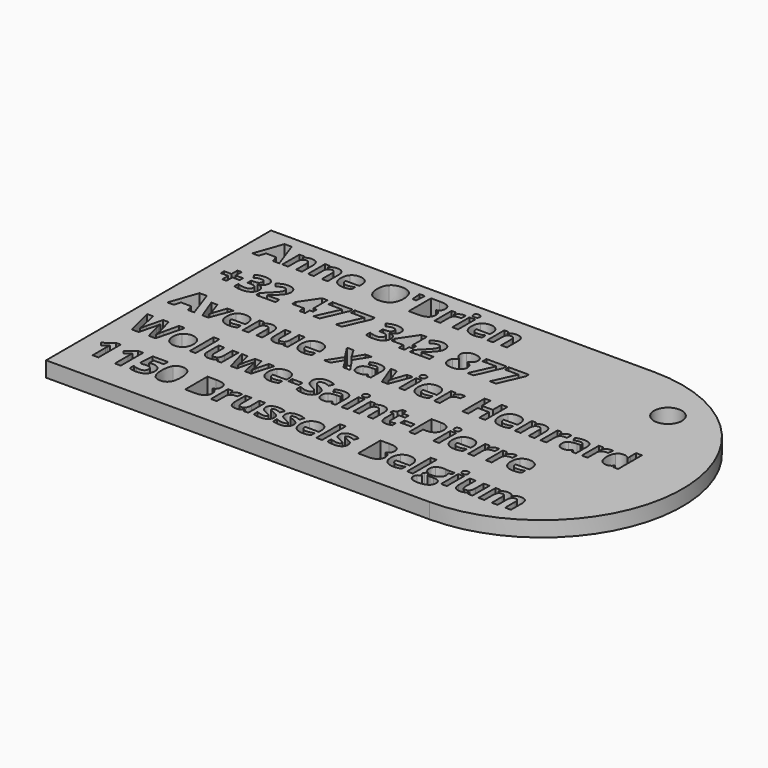
from build123d import *

# Parameters (mm, degrees)
F0_W     = 1.1374782986
F0_H     = 5.8043619792
F0_W_2   = 2.0028211806
F0_H_2   = 0.9321831597
F0_H_3   = 4.1703559028
F0_R     = 2.7240159919
F1_DEPTH = 3


with BuildPart() as f1:
    # F0 (on Top) → F1 (new body)
    with BuildSketch(Plane.XY):
        with BuildLine():
            Line((57.442756952, 2.8984979283), (-17.557243048, 2.8984979283))
            Line((-17.557243048, 2.8984979283), (-17.557243048, -52.1015020717))
            Line((-17.557243048, -52.1015020717), (57.442756952, -52.1015020717))
            ThreePointArc((57.442756952, -52.1015020717), (84.942756952, -24.6015020717), (57.442756952, 2.8984979283))
        make_face()
        with BuildLine():
            Line((-11.9014270758, -40.9091559052), (-11.9014270758, -46.362606426))
            Line((-11.9014270758, -46.362606426), (-13.0544218675, -46.362606426))
            Line((-13.0544218675, -46.362606426), (-13.0544218675, -43.2067904538))
            Line((-13.0544218675, -43.2067904538), (-13.0424861036, -42.688778301))
            Line((-13.0424861036, -42.688778301), (-13.0245824578, -42.1218295163))
            add(Edge.make_bspline(
                [(-13.0245824578, -42.1218295163), (-13.3110407911, -42.4082878496), (-13.4232369717, -42.4978060788)],
                knots=[0, 0, 0, 1, 1, 1], degree=2))
            Line((-13.4232369717, -42.4978060788), (-14.0498645758, -43.0014953149))
            Line((-14.0498645758, -43.0014953149), (-14.606071173, -42.308027433))
            Line((-14.606071173, -42.308027433), (-12.8491267286, -40.9091559052))
            Line((-12.8491267286, -40.9091559052), (-11.9014270758, -40.9091559052))
        make_face(mode=Mode.SUBTRACT)
        with BuildLine():
            Line((-7.5412925272, -40.9091559052), (-7.5412925272, -46.362606426))
            Line((-7.5412925272, -46.362606426), (-8.6942873189, -46.362606426))
            Line((-8.6942873189, -46.362606426), (-8.6942873189, -43.2067904538))
            Line((-8.6942873189, -43.2067904538), (-8.682351555, -42.688778301))
            Line((-8.682351555, -42.688778301), (-8.6644479092, -42.1218295163))
            add(Edge.make_bspline(
                [(-8.6644479092, -42.1218295163), (-8.9509062425, -42.4082878496), (-9.063102423, -42.4978060788)],
                knots=[0, 0, 0, 1, 1, 1], degree=2))
            Line((-9.063102423, -42.4978060788), (-9.6897300272, -43.0014953149))
            Line((-9.6897300272, -43.0014953149), (-10.2459366244, -42.308027433))
            Line((-10.2459366244, -42.308027433), (-8.48899218, -40.9091559052))
            Line((-8.48899218, -40.9091559052), (-7.5412925272, -40.9091559052))
        make_face(mode=Mode.SUBTRACT)
        with BuildLine():
            add(Edge.make_bspline(
                [(-4.6098689161, -42.931074308), (-4.3818958258, -42.8785569468), (-4.0465008605, -42.8785569468)],
                knots=[0, 0, 0, 1, 1, 1], degree=2))
            add(Edge.make_bspline(
                [(-4.0465008605, -42.8785569468), (-3.2563532911, -42.8785569468), (-2.7878745585, -43.3225673635)],
                knots=[0, 0, 0, 1, 1, 1], degree=2))
            add(Edge.make_bspline(
                [(-2.7878745585, -43.3225673635), (-2.3193958258, -43.7665777802), (-2.3193958258, -44.5388217038)],
                knots=[0, 0, 0, 1, 1, 1], degree=2))
            add(Edge.make_bspline(
                [(-2.3193958258, -44.5388217038), (-2.3193958258, -45.4519076413), (-2.8827638814, -45.9448546899)],
                knots=[0, 0, 0, 1, 1, 1], degree=2))
            add(Edge.make_bspline(
                [(-2.8827638814, -45.9448546899), (-3.4461319369, -46.4378017385), (-4.4940920064, -46.4378017385)],
                knots=[0, 0, 0, 1, 1, 1], degree=2))
            add(Edge.make_bspline(
                [(-4.4940920064, -46.4378017385), (-5.4047907911, -46.4378017385), (-5.9633845411, -46.1429883705)],
                knots=[0, 0, 0, 1, 1, 1], degree=2))
            Line((-5.9633845411, -46.1429883705), (-5.9633845411, -45.1463520857))
            add(Edge.make_bspline(
                [(-5.9633845411, -45.1463520857), (-5.6697647494, -45.3027105927), (-5.2776749057, -45.401777433)],
                knots=[0, 0, 0, 1, 1, 1], degree=2))
            add(Edge.make_bspline(
                [(-5.2776749057, -45.401777433), (-4.8855850619, -45.5008442732), (-4.53586718, -45.5008442732)],
                knots=[0, 0, 0, 1, 1, 1], degree=2))
            add(Edge.make_bspline(
                [(-4.53586718, -45.5008442732), (-3.4795520758, -45.5008442732), (-3.4795520758, -44.6355013913)],
                knots=[0, 0, 0, 1, 1, 1], degree=2))
            add(Edge.make_bspline(
                [(-3.4795520758, -44.6355013913), (-3.4795520758, -43.8107401066), (-4.572868048, -43.8107401066)],
                knots=[0, 0, 0, 1, 1, 1], degree=2))
            add(Edge.make_bspline(
                [(-4.572868048, -43.8107401066), (-4.7698081522, -43.8107401066), (-5.00852343, -43.8501281274)],
                knots=[0, 0, 0, 1, 1, 1], degree=2))
            add(Edge.make_bspline(
                [(-5.00852343, -43.8501281274), (-5.2472387078, -43.8895161482), (-5.3964357564, -43.934872051)],
                knots=[0, 0, 0, 1, 1, 1], degree=2))
            Line((-5.3964357564, -43.934872051), (-5.8559626661, -43.6878017385))
            Line((-5.8559626661, -43.6878017385), (-5.6506675272, -40.9091559052))
            Line((-5.6506675272, -40.9091559052), (-2.6929852355, -40.9091559052))
            Line((-2.6929852355, -40.9091559052), (-2.6929852355, -41.8866949677))
            Line((-2.6929852355, -41.8866949677), (-4.6397083258, -41.8866949677))
            Line((-4.6397083258, -41.8866949677), (-4.7399687425, -42.9573329885))
            Line((-4.7399687425, -42.9573329885), (-4.6098689161, -42.931074308))
        make_face(mode=Mode.SUBTRACT)
        with BuildLine():
            add(Edge.make_bspline(
                [(1.6283580804, -41.5393642385), (2.1111597297, -42.2555100718), (2.1111597297, -43.6364779538)],
                knots=[0, 0, 0, 1, 1, 1], degree=2))
            add(Edge.make_bspline(
                [(2.1111597297, -43.6364779538), (2.1111597297, -45.0639953149), (1.6432777853, -45.7508985267)],
                knots=[0, 0, 0, 1, 1, 1], degree=2))
            add(Edge.make_bspline(
                [(1.6432777853, -45.7508985267), (1.1753958408, -46.4378017385), (0.2014375075, -46.4378017385)],
                knots=[0, 0, 0, 1, 1, 1], degree=2))
            add(Edge.make_bspline(
                [(0.2014375075, -46.4378017385), (-0.7426814161, -46.4378017385), (-1.2219023362, -45.7288173635)],
                knots=[0, 0, 0, 1, 1, 1], degree=2))
            add(Edge.make_bspline(
                [(-1.2219023362, -45.7288173635), (-1.7011232564, -45.0198329885), (-1.7011232564, -43.6364779538)],
                knots=[0, 0, 0, 1, 1, 1], degree=2))
            add(Edge.make_bspline(
                [(-1.7011232564, -43.6364779538), (-1.7011232564, -42.1922505232), (-1.2344348883, -41.5077344642)],
                knots=[0, 0, 0, 1, 1, 1], degree=2))
            add(Edge.make_bspline(
                [(-1.2344348883, -41.5077344642), (-0.7677465203, -40.8232184052), (0.2014375075, -40.8232184052)],
                knots=[0, 0, 0, 1, 1, 1], degree=2))
            add(Edge.make_bspline(
                [(0.2014375075, -40.8232184052), (1.1455564311, -40.8232184052), (1.6283580804, -41.5393642385)],
                knots=[0, 0, 0, 1, 1, 1], degree=2))
        make_face(mode=Mode.SUBTRACT)
        with BuildLine():
            Line((5.0545191047, -46.362606426), (5.0545191047, -40.9091559052))
            Line((5.0545191047, -40.9091559052), (6.7517847297, -40.9091559052))
            add(Edge.make_bspline(
                [(6.7517847297, -40.9091559052), (7.9119409797, -40.9091559052), (8.4359210145, -41.2391797767)],
                knots=[0, 0, 0, 1, 1, 1], degree=2))
            add(Edge.make_bspline(
                [(8.4359210145, -41.2391797767), (8.9599010492, -41.5692036482), (8.9599010492, -42.2889302107)],
                knots=[0, 0, 0, 1, 1, 1], degree=2))
            add(Edge.make_bspline(
                [(8.9599010492, -42.2889302107), (8.9599010492, -42.7782965302), (8.7307343825, -43.0916103323)],
                knots=[0, 0, 0, 1, 1, 1], degree=2))
            add(Edge.make_bspline(
                [(8.7307343825, -43.0916103323), (8.5015677158, -43.4049241343), (8.1208168478, -43.468183683)],
                knots=[0, 0, 0, 1, 1, 1], degree=2))
            Line((8.1208168478, -43.468183683), (8.1208168478, -43.505184551))
            add(Edge.make_bspline(
                [(8.1208168478, -43.505184551), (8.6388290006, -43.6209614607), (8.8685924554, -43.937855992)],
                knots=[0, 0, 0, 1, 1, 1], degree=2))
            add(Edge.make_bspline(
                [(8.8685924554, -43.937855992), (9.0983559103, -44.2547505232), (9.0983559103, -44.7811177107)],
                knots=[0, 0, 0, 1, 1, 1], degree=2))
            add(Edge.make_bspline(
                [(9.0983559103, -44.7811177107), (9.0983559103, -45.5271029538), (8.5588593825, -45.9448546899)],
                knots=[0, 0, 0, 1, 1, 1], degree=2))
            add(Edge.make_bspline(
                [(8.5588593825, -45.9448546899), (8.0193628547, -46.362606426), (7.0943411533, -46.362606426)],
                knots=[0, 0, 0, 1, 1, 1], degree=2))
            Line((7.0943411533, -46.362606426), (5.0545191047, -46.362606426))
        make_face(mode=Mode.SUBTRACT)
        with BuildLine():
            add(Edge.make_bspline(
                [(11.7069171082, -42.3289150198), (12.0369409797, -42.114668058), (12.4248533061, -42.114668058)],
                knots=[0, 0, 0, 1, 1, 1], degree=2))
            add(Edge.make_bspline(
                [(12.4248533061, -42.114668058), (12.6564071256, -42.114668058), (12.8091849033, -42.1480881968)],
                knots=[0, 0, 0, 1, 1, 1], degree=2))
            Line((12.8091849033, -42.1480881968), (12.7232474033, -43.2139519121))
            add(Edge.make_bspline(
                [(12.7232474033, -43.2139519121), (12.5847925422, -43.1769510441), (12.3878524381, -43.1769510441)],
                knots=[0, 0, 0, 1, 1, 1], degree=2))
            add(Edge.make_bspline(
                [(12.3878524381, -43.1769510441), (11.8435816047, -43.1769510441), (11.5392196256, -43.4568447073)],
                knots=[0, 0, 0, 1, 1, 1], degree=2))
            add(Edge.make_bspline(
                [(11.5392196256, -43.4568447073), (11.2348576464, -43.7367383705), (11.2348576464, -44.2404276066)],
                knots=[0, 0, 0, 1, 1, 1], degree=2))
            Line((11.2348576464, -44.2404276066), (11.2348576464, -46.362606426))
            Line((11.2348576464, -46.362606426), (10.0973793478, -46.362606426))
            Line((10.0973793478, -46.362606426), (10.0973793478, -42.1922505232))
            Line((10.0973793478, -42.1922505232), (10.9591415006, -42.1922505232))
            Line((10.9591415006, -42.1922505232), (11.1274357714, -42.8940734399))
            Line((11.1274357714, -42.8940734399), (11.1823402853, -42.8940734399))
            add(Edge.make_bspline(
                [(11.1823402853, -42.8940734399), (11.3768932367, -42.5431619816), (11.7069171082, -42.3289150198)],
                knots=[0, 0, 0, 1, 1, 1], degree=2))
        make_face(mode=Mode.SUBTRACT)
        with BuildLine():
            Line((17.3925182367, -46.362606426), (16.5200138964, -46.362606426))
            Line((16.5200138964, -46.362606426), (16.3672361186, -45.8290777802))
            Line((16.3672361186, -45.8290777802), (16.3075572992, -45.8290777802))
            add(Edge.make_bspline(
                [(16.3075572992, -45.8290777802), (16.1249401117, -46.1203104191), (15.7889483582, -46.2790560788)],
                knots=[0, 0, 0, 1, 1, 1], degree=2))
            add(Edge.make_bspline(
                [(15.7889483582, -46.2790560788), (15.4529566047, -46.4378017385), (15.0244626811, -46.4378017385)],
                knots=[0, 0, 0, 1, 1, 1], degree=2))
            add(Edge.make_bspline(
                [(15.0244626811, -46.4378017385), (14.2892196256, -46.4378017385), (13.916227004, -46.0439215302)],
                knots=[0, 0, 0, 1, 1, 1], degree=2))
            add(Edge.make_bspline(
                [(13.916227004, -46.0439215302), (13.5432343825, -45.6500413218), (13.5432343825, -44.9112175371)],
                knots=[0, 0, 0, 1, 1, 1], degree=2))
            Line((13.5432343825, -44.9112175371), (13.5432343825, -42.1922505232))
            Line((13.5432343825, -42.1922505232), (14.6807126811, -42.1922505232))
            Line((14.6807126811, -42.1922505232), (14.6807126811, -44.628339933))
            add(Edge.make_bspline(
                [(14.6807126811, -44.628339933), (14.6807126811, -45.079511808), (14.8412487054, -45.3050977455)],
                knots=[0, 0, 0, 1, 1, 1], degree=2))
            add(Edge.make_bspline(
                [(14.8412487054, -45.3050977455), (15.0017847297, -45.530683683), (15.3526961881, -45.530683683)],
                knots=[0, 0, 0, 1, 1, 1], degree=2))
            add(Edge.make_bspline(
                [(15.3526961881, -45.530683683), (15.8301267436, -45.530683683), (16.0425833408, -45.2119987871)],
                knots=[0, 0, 0, 1, 1, 1], degree=2))
            add(Edge.make_bspline(
                [(16.0425833408, -45.2119987871), (16.2550399381, -44.8933138913), (16.2550399381, -44.1544901066)],
                knots=[0, 0, 0, 1, 1, 1], degree=2))
            Line((16.2550399381, -44.1544901066), (16.2550399381, -42.1922505232))
            Line((16.2550399381, -42.1922505232), (17.3925182367, -42.1922505232))
            Line((17.3925182367, -42.1922505232), (17.3925182367, -46.362606426))
        make_face(mode=Mode.SUBTRACT)
        with BuildLine():
            add(Edge.make_bspline(
                [(21.3874184103, -44.5907422767), (21.4960338617, -44.8145378496), (21.4960338617, -45.1236741343)],
                knots=[0, 0, 0, 1, 1, 1], degree=2))
            add(Edge.make_bspline(
                [(21.4960338617, -45.1236741343), (21.4960338617, -45.7658182316), (21.0502330804, -46.101809985)],
                knots=[0, 0, 0, 1, 1, 1], degree=2))
            add(Edge.make_bspline(
                [(21.0502330804, -46.101809985), (20.6044322992, -46.4378017385), (19.7164114658, -46.4378017385)],
                knots=[0, 0, 0, 1, 1, 1], degree=2))
            add(Edge.make_bspline(
                [(19.7164114658, -46.4378017385), (19.2616588617, -46.4378017385), (18.9405868131, -46.3757357663)],
                knots=[0, 0, 0, 1, 1, 1], degree=2))
            add(Edge.make_bspline(
                [(18.9405868131, -46.3757357663), (18.6195147645, -46.3136697941), (18.3402178895, -46.1943121552)],
                knots=[0, 0, 0, 1, 1, 1], degree=2))
            Line((18.3402178895, -46.1943121552), (18.3402178895, -45.2549675371))
            add(Edge.make_bspline(
                [(18.3402178895, -45.2549675371), (18.6565156325, -45.4041645857), (19.05397657, -45.5050217906)],
                knots=[0, 0, 0, 1, 1, 1], degree=2))
            add(Edge.make_bspline(
                [(19.05397657, -45.5050217906), (19.4514375075, -45.6058789955), (19.7534123339, -45.6058789955)],
                knots=[0, 0, 0, 1, 1, 1], degree=2))
            add(Edge.make_bspline(
                [(19.7534123339, -45.6058789955), (20.3728784797, -45.6058789955), (20.3728784797, -45.2478060788)],
                knots=[0, 0, 0, 1, 1, 1], degree=2))
            add(Edge.make_bspline(
                [(20.3728784797, -45.2478060788), (20.3728784797, -45.1129319468), (20.2905217089, -45.0287848114)],
                knots=[0, 0, 0, 1, 1, 1], degree=2))
            add(Edge.make_bspline(
                [(20.2905217089, -45.0287848114), (20.2081649381, -44.944637676), (20.0070473165, -44.8384093774)],
                knots=[0, 0, 0, 1, 1, 1], degree=2))
            add(Edge.make_bspline(
                [(20.0070473165, -44.8384093774), (19.805929695, -44.7321810788), (19.4705347297, -44.5913390649)],
                knots=[0, 0, 0, 1, 1, 1], degree=2))
            add(Edge.make_bspline(
                [(19.4705347297, -44.5913390649), (18.989523445, -44.3896246552), (18.7633407193, -44.2177496552)],
                knots=[0, 0, 0, 1, 1, 1], degree=2))
            add(Edge.make_bspline(
                [(18.7633407193, -44.2177496552), (18.5371579936, -44.0458746552), (18.4351072124, -43.8238694468)],
                knots=[0, 0, 0, 1, 1, 1], degree=2))
            add(Edge.make_bspline(
                [(18.4351072124, -43.8238694468), (18.3330564311, -43.6018642385), (18.3330564311, -43.2784050371)],
                knots=[0, 0, 0, 1, 1, 1], degree=2))
            add(Edge.make_bspline(
                [(18.3330564311, -43.2784050371), (18.3330564311, -42.7221984399), (18.7633407193, -42.4184332489)],
                knots=[0, 0, 0, 1, 1, 1], degree=2))
            add(Edge.make_bspline(
                [(18.7633407193, -42.4184332489), (19.1936250075, -42.114668058), (19.9849661533, -42.114668058)],
                knots=[0, 0, 0, 1, 1, 1], degree=2))
            add(Edge.make_bspline(
                [(19.9849661533, -42.114668058), (20.7381128547, -42.114668058), (21.4506779589, -42.4429015649)],
                knots=[0, 0, 0, 1, 1, 1], degree=2))
            Line((21.4506779589, -42.4429015649), (21.1081215353, -43.2628885441))
            add(Edge.make_bspline(
                [(21.1081215353, -43.2628885441), (20.794210945, -43.1292079885), (20.5220755283, -43.0432704885)],
                knots=[0, 0, 0, 1, 1, 1], degree=2))
            add(Edge.make_bspline(
                [(20.5220755283, -43.0432704885), (20.2499401117, -42.9573329885), (19.9658689311, -42.9573329885)],
                knots=[0, 0, 0, 1, 1, 1], degree=2))
            add(Edge.make_bspline(
                [(19.9658689311, -42.9573329885), (19.462179695, -42.9573329885), (19.462179695, -43.2294684052)],
                knots=[0, 0, 0, 1, 1, 1], degree=2))
            add(Edge.make_bspline(
                [(19.462179695, -43.2294684052), (19.462179695, -43.382246183), (19.6245060839, -43.4944423635)],
                knots=[0, 0, 0, 1, 1, 1], degree=2))
            add(Edge.make_bspline(
                [(19.6245060839, -43.4944423635), (19.7868324728, -43.6066385441), (20.3358776117, -43.8262565996)],
                knots=[0, 0, 0, 1, 1, 1], degree=2))
            add(Edge.make_bspline(
                [(20.3358776117, -43.8262565996), (20.8240503547, -44.0243902802), (21.0514266568, -44.195668492)],
                knots=[0, 0, 0, 1, 1, 1], degree=2))
            add(Edge.make_bspline(
                [(21.0514266568, -44.195668492), (21.2788029589, -44.3669467038), (21.3874184103, -44.5907422767)],
                knots=[0, 0, 0, 1, 1, 1], degree=2))
        make_face(mode=Mode.SUBTRACT)
        with BuildLine():
            add(Edge.make_bspline(
                [(25.1841849033, -44.5907422767), (25.2928003547, -44.8145378496), (25.2928003547, -45.1236741343)],
                knots=[0, 0, 0, 1, 1, 1], degree=2))
            add(Edge.make_bspline(
                [(25.2928003547, -45.1236741343), (25.2928003547, -45.7658182316), (24.8469995735, -46.101809985)],
                knots=[0, 0, 0, 1, 1, 1], degree=2))
            add(Edge.make_bspline(
                [(24.8469995735, -46.101809985), (24.4011987922, -46.4378017385), (23.5131779589, -46.4378017385)],
                knots=[0, 0, 0, 1, 1, 1], degree=2))
            add(Edge.make_bspline(
                [(23.5131779589, -46.4378017385), (23.0584253547, -46.4378017385), (22.7373533061, -46.3757357663)],
                knots=[0, 0, 0, 1, 1, 1], degree=2))
            add(Edge.make_bspline(
                [(22.7373533061, -46.3757357663), (22.4162812575, -46.3136697941), (22.1369843825, -46.1943121552)],
                knots=[0, 0, 0, 1, 1, 1], degree=2))
            Line((22.1369843825, -46.1943121552), (22.1369843825, -45.2549675371))
            add(Edge.make_bspline(
                [(22.1369843825, -45.2549675371), (22.4532821256, -45.4041645857), (22.8507430631, -45.5050217906)],
                knots=[0, 0, 0, 1, 1, 1], degree=2))
            add(Edge.make_bspline(
                [(22.8507430631, -45.5050217906), (23.2482040006, -45.6058789955), (23.550178827, -45.6058789955)],
                knots=[0, 0, 0, 1, 1, 1], degree=2))
            add(Edge.make_bspline(
                [(23.550178827, -45.6058789955), (24.1696449728, -45.6058789955), (24.1696449728, -45.2478060788)],
                knots=[0, 0, 0, 1, 1, 1], degree=2))
            add(Edge.make_bspline(
                [(24.1696449728, -45.2478060788), (24.1696449728, -45.1129319468), (24.087288202, -45.0287848114)],
                knots=[0, 0, 0, 1, 1, 1], degree=2))
            add(Edge.make_bspline(
                [(24.087288202, -45.0287848114), (24.0049314311, -44.944637676), (23.8038138096, -44.8384093774)],
                knots=[0, 0, 0, 1, 1, 1], degree=2))
            add(Edge.make_bspline(
                [(23.8038138096, -44.8384093774), (23.6026961881, -44.7321810788), (23.2673012228, -44.5913390649)],
                knots=[0, 0, 0, 1, 1, 1], degree=2))
            add(Edge.make_bspline(
                [(23.2673012228, -44.5913390649), (22.7862899381, -44.3896246552), (22.5601072124, -44.2177496552)],
                knots=[0, 0, 0, 1, 1, 1], degree=2))
            add(Edge.make_bspline(
                [(22.5601072124, -44.2177496552), (22.3339244867, -44.0458746552), (22.2318737054, -43.8238694468)],
                knots=[0, 0, 0, 1, 1, 1], degree=2))
            add(Edge.make_bspline(
                [(22.2318737054, -43.8238694468), (22.1298229242, -43.6018642385), (22.1298229242, -43.2784050371)],
                knots=[0, 0, 0, 1, 1, 1], degree=2))
            add(Edge.make_bspline(
                [(22.1298229242, -43.2784050371), (22.1298229242, -42.7221984399), (22.5601072124, -42.4184332489)],
                knots=[0, 0, 0, 1, 1, 1], degree=2))
            add(Edge.make_bspline(
                [(22.5601072124, -42.4184332489), (22.9903915006, -42.114668058), (23.7817326464, -42.114668058)],
                knots=[0, 0, 0, 1, 1, 1], degree=2))
            add(Edge.make_bspline(
                [(23.7817326464, -42.114668058), (24.5348793478, -42.114668058), (25.247444452, -42.4429015649)],
                knots=[0, 0, 0, 1, 1, 1], degree=2))
            Line((25.247444452, -42.4429015649), (24.9048880283, -43.2628885441))
            add(Edge.make_bspline(
                [(24.9048880283, -43.2628885441), (24.5909774381, -43.1292079885), (24.3188420214, -43.0432704885)],
                knots=[0, 0, 0, 1, 1, 1], degree=2))
            add(Edge.make_bspline(
                [(24.3188420214, -43.0432704885), (24.0467066047, -42.9573329885), (23.7626354242, -42.9573329885)],
                knots=[0, 0, 0, 1, 1, 1], degree=2))
            add(Edge.make_bspline(
                [(23.7626354242, -42.9573329885), (23.2589461881, -42.9573329885), (23.2589461881, -43.2294684052)],
                knots=[0, 0, 0, 1, 1, 1], degree=2))
            add(Edge.make_bspline(
                [(23.2589461881, -43.2294684052), (23.2589461881, -43.382246183), (23.421272577, -43.4944423635)],
                knots=[0, 0, 0, 1, 1, 1], degree=2))
            add(Edge.make_bspline(
                [(23.421272577, -43.4944423635), (23.5835989658, -43.6066385441), (24.1326441047, -43.8262565996)],
                knots=[0, 0, 0, 1, 1, 1], degree=2))
            add(Edge.make_bspline(
                [(24.1326441047, -43.8262565996), (24.6208168478, -44.0243902802), (24.8481931499, -44.195668492)],
                knots=[0, 0, 0, 1, 1, 1], degree=2))
            add(Edge.make_bspline(
                [(24.8481931499, -44.195668492), (25.075569452, -44.3669467038), (25.1841849033, -44.5907422767)],
                knots=[0, 0, 0, 1, 1, 1], degree=2))
        make_face(mode=Mode.SUBTRACT)
        with BuildLine():
            add(Edge.make_bspline(
                [(28.8950138964, -46.3649935788), (28.556038202, -46.4378017385), (28.0666718825, -46.4378017385)],
                knots=[0, 0, 0, 1, 1, 1], degree=2))
            add(Edge.make_bspline(
                [(28.0666718825, -46.4378017385), (27.0604869867, -46.4378017385), (26.493538202, -45.8815951413)],
                knots=[0, 0, 0, 1, 1, 1], degree=2))
            add(Edge.make_bspline(
                [(26.493538202, -45.8815951413), (25.9265894172, -45.3253885441), (25.9265894172, -44.3072678843)],
                knots=[0, 0, 0, 1, 1, 1], degree=2))
            add(Edge.make_bspline(
                [(25.9265894172, -44.3072678843), (25.9265894172, -43.2593078149), (26.450569452, -42.6869879364)],
                knots=[0, 0, 0, 1, 1, 1], degree=2))
            add(Edge.make_bspline(
                [(26.450569452, -42.6869879364), (26.9745494867, -42.114668058), (27.8995711881, -42.114668058)],
                knots=[0, 0, 0, 1, 1, 1], degree=2))
            add(Edge.make_bspline(
                [(27.8995711881, -42.114668058), (28.7828177158, -42.114668058), (29.2751679763, -42.6177605059)],
                knots=[0, 0, 0, 1, 1, 1], degree=2))
            add(Edge.make_bspline(
                [(29.2751679763, -42.6177605059), (29.7675182367, -43.1208529538), (29.7675182367, -44.0088737871)],
                knots=[0, 0, 0, 1, 1, 1], degree=2))
            Line((29.7675182367, -44.0088737871), (29.7675182367, -44.5614996552))
            Line((29.7675182367, -44.5614996552), (27.0783906325, -44.5614996552))
            add(Edge.make_bspline(
                [(27.0783906325, -44.5614996552), (27.0974878547, -45.0460916691), (27.3660425422, -45.3182270857)],
                knots=[0, 0, 0, 1, 1, 1], degree=2))
            add(Edge.make_bspline(
                [(27.3660425422, -45.3182270857), (27.6345972297, -45.5903625024), (28.1191892436, -45.5903625024)],
                knots=[0, 0, 0, 1, 1, 1], degree=2))
            add(Edge.make_bspline(
                [(28.1191892436, -45.5903625024), (28.4963593825, -45.5903625024), (28.8317543478, -45.5121832489)],
                knots=[0, 0, 0, 1, 1, 1], degree=2))
            add(Edge.make_bspline(
                [(28.8317543478, -45.5121832489), (29.1671493131, -45.4340039955), (29.5323836881, -45.2621289955)],
                knots=[0, 0, 0, 1, 1, 1], degree=2))
            Line((29.5323836881, -45.2621289955), (29.5323836881, -46.1429883705))
            add(Edge.make_bspline(
                [(29.5323836881, -46.1429883705), (29.2339895908, -46.2921854191), (28.8950138964, -46.3649935788)],
                knots=[0, 0, 0, 1, 1, 1], degree=2))
        make_face(mode=Mode.SUBTRACT)
        with Locations((31.2612790874, -43.4604254364)):
            Rectangle(F0_W, F0_H, mode=Mode.SUBTRACT)
        with BuildLine():
            Line((-7.6713923536, -30.5202670163), (-9.0595216939, -35.9737175371))
            Line((-9.0595216939, -35.9737175371), (-10.3760364508, -35.9737175371))
            Line((-10.3760364508, -35.9737175371), (-11.1148602355, -33.1091342038))
            add(Edge.make_bspline(
                [(-11.1148602355, -33.1091342038), (-11.1554418328, -32.956356426), (-11.254508673, -32.4771355059)],
                knots=[0, 0, 0, 1, 1, 1], degree=2))
            add(Edge.make_bspline(
                [(-11.254508673, -32.4771355059), (-11.3535755133, -31.9979145857), (-11.36789843, -31.8332010441)],
                knots=[0, 0, 0, 1, 1, 1], degree=2))
            add(Edge.make_bspline(
                [(-11.36789843, -31.8332010441), (-11.3905763814, -32.0349154538), (-11.4800946105, -32.480716235)],
                knots=[0, 0, 0, 1, 1, 1], degree=2))
            add(Edge.make_bspline(
                [(-11.4800946105, -32.480716235), (-11.5696128397, -32.9265170163), (-11.6185494717, -33.1162956621)],
                knots=[0, 0, 0, 1, 1, 1], degree=2))
            Line((-11.6185494717, -33.1162956621), (-12.3525989508, -35.9737175371))
            Line((-12.3525989508, -35.9737175371), (-13.6655329786, -35.9737175371))
            Line((-13.6655329786, -35.9737175371), (-15.057243048, -30.5202670163))
            Line((-15.057243048, -30.5202670163), (-13.9197647494, -30.5202670163))
            Line((-13.9197647494, -30.5202670163), (-13.2215225619, -33.4970465302))
            add(Edge.make_bspline(
                [(-13.2215225619, -33.4970465302), (-13.0389053744, -34.3218078149), (-12.95774218, -34.9257574677)],
                knots=[0, 0, 0, 1, 1, 1], degree=2))
            add(Edge.make_bspline(
                [(-12.95774218, -34.9257574677), (-12.9350642286, -34.7133008705), (-12.8544978224, -34.2675000892)],
                knots=[0, 0, 0, 1, 1, 1], degree=2))
            add(Edge.make_bspline(
                [(-12.8544978224, -34.2675000892), (-12.7739314161, -33.821699308), (-12.7035104092, -33.5758225718)],
                knots=[0, 0, 0, 1, 1, 1], degree=2))
            Line((-12.7035104092, -33.5758225718), (-11.9085885342, -30.5202670163))
            Line((-11.9085885342, -30.5202670163), (-10.8164661383, -30.5202670163))
            Line((-10.8164661383, -30.5202670163), (-10.0215442633, -33.5758225718))
            add(Edge.make_bspline(
                [(-10.0215442633, -33.5758225718), (-9.9690269022, -33.7799241343), (-9.8908476487, -34.2018533878)],
                knots=[0, 0, 0, 1, 1, 1], degree=2))
            add(Edge.make_bspline(
                [(-9.8908476487, -34.2018533878), (-9.8126683953, -34.6237826413), (-9.772086798, -34.9257574677)],
                knots=[0, 0, 0, 1, 1, 1], degree=2))
            add(Edge.make_bspline(
                [(-9.772086798, -34.9257574677), (-9.73508593, -34.6345248288), (-9.6527291592, -34.2000630232)],
                knots=[0, 0, 0, 1, 1, 1], degree=2))
            add(Edge.make_bspline(
                [(-9.6527291592, -34.2000630232), (-9.5703723883, -33.7656012177), (-9.5035321105, -33.4970465302)],
                knots=[0, 0, 0, 1, 1, 1], degree=2))
            Line((-9.5035321105, -33.4970465302), (-8.8100642286, -30.5202670163))
            Line((-8.8100642286, -30.5202670163), (-7.6713923536, -30.5202670163))
        make_face(mode=Mode.SUBTRACT)
        with BuildLine():
            add(Edge.make_bspline(
                [(-3.5308758605, -32.7361415823), (-3.2849991244, -33.2249111135), (-3.2849991244, -33.8813781274)],
                knots=[0, 0, 0, 1, 1, 1], degree=2))
            add(Edge.make_bspline(
                [(-3.2849991244, -33.8813781274), (-3.2849991244, -34.8994987871), (-3.8221084994, -35.4742058184)],
                knots=[0, 0, 0, 1, 1, 1], degree=2))
            add(Edge.make_bspline(
                [(-3.8221084994, -35.4742058184), (-4.3592178744, -36.0489128496), (-5.3176597147, -36.0489128496)],
                knots=[0, 0, 0, 1, 1, 1], degree=2))
            add(Edge.make_bspline(
                [(-5.3176597147, -36.0489128496), (-5.9180286383, -36.0489128496), (-6.3769587599, -35.7857292559)],
                knots=[0, 0, 0, 1, 1, 1], degree=2))
            add(Edge.make_bspline(
                [(-6.3769587599, -35.7857292559), (-6.8358888814, -35.5225456621), (-7.0817656175, -35.0301954017)],
                knots=[0, 0, 0, 1, 1, 1], degree=2))
            add(Edge.make_bspline(
                [(-7.0817656175, -35.0301954017), (-7.3276423536, -34.5378451413), (-7.3276423536, -33.8813781274)],
                knots=[0, 0, 0, 1, 1, 1], degree=2))
            add(Edge.make_bspline(
                [(-7.3276423536, -33.8813781274), (-7.3276423536, -32.8596767385), (-6.794710496, -32.2927279538)],
                knots=[0, 0, 0, 1, 1, 1], degree=2))
            add(Edge.make_bspline(
                [(-6.794710496, -32.2927279538), (-6.2617786383, -31.7257791691), (-5.2949817633, -31.7257791691)],
                knots=[0, 0, 0, 1, 1, 1], degree=2))
            add(Edge.make_bspline(
                [(-5.2949817633, -31.7257791691), (-4.6946128397, -31.7257791691), (-4.2356827182, -31.98657561)],
                knots=[0, 0, 0, 1, 1, 1], degree=2))
            add(Edge.make_bspline(
                [(-4.2356827182, -31.98657561), (-3.7767525967, -32.247372051), (-3.5308758605, -32.7361415823)],
                knots=[0, 0, 0, 1, 1, 1], degree=2))
        make_face(mode=Mode.SUBTRACT)
        with Locations((-1.7757217807, -33.0715365475)):
            Rectangle(F0_W, F0_H, mode=Mode.SUBTRACT)
        with BuildLine():
            Line((3.8131996603, -35.9737175371), (2.94069532, -35.9737175371))
            Line((2.94069532, -35.9737175371), (2.7879175422, -35.4401888913))
            Line((2.7879175422, -35.4401888913), (2.7282387228, -35.4401888913))
            add(Edge.make_bspline(
                [(2.7282387228, -35.4401888913), (2.5456215353, -35.7314215302), (2.2096297818, -35.8901671899)],
                knots=[0, 0, 0, 1, 1, 1], degree=2))
            add(Edge.make_bspline(
                [(2.2096297818, -35.8901671899), (1.8736380283, -36.0489128496), (1.4451441047, -36.0489128496)],
                knots=[0, 0, 0, 1, 1, 1], degree=2))
            add(Edge.make_bspline(
                [(1.4451441047, -36.0489128496), (0.7099010492, -36.0489128496), (0.3369084276, -35.6550326413)],
                knots=[0, 0, 0, 1, 1, 1], degree=2))
            add(Edge.make_bspline(
                [(0.3369084276, -35.6550326413), (-0.0360841939, -35.261152433), (-0.0360841939, -34.5223286482)],
                knots=[0, 0, 0, 1, 1, 1], degree=2))
            Line((-0.0360841939, -34.5223286482), (-0.0360841939, -31.8033616343))
            Line((-0.0360841939, -31.8033616343), (1.1013941047, -31.8033616343))
            Line((1.1013941047, -31.8033616343), (1.1013941047, -34.2394510441))
            add(Edge.make_bspline(
                [(1.1013941047, -34.2394510441), (1.1013941047, -34.6906229191), (1.261930129, -34.9162088566)],
                knots=[0, 0, 0, 1, 1, 1], degree=2))
            add(Edge.make_bspline(
                [(1.261930129, -34.9162088566), (1.4224661533, -35.1417947941), (1.7733776117, -35.1417947941)],
                knots=[0, 0, 0, 1, 1, 1], degree=2))
            add(Edge.make_bspline(
                [(1.7733776117, -35.1417947941), (2.2508081672, -35.1417947941), (2.4632647645, -34.8231098982)],
                knots=[0, 0, 0, 1, 1, 1], degree=2))
            add(Edge.make_bspline(
                [(2.4632647645, -34.8231098982), (2.6757213617, -34.5044250024), (2.6757213617, -33.7656012177)],
                knots=[0, 0, 0, 1, 1, 1], degree=2))
            Line((2.6757213617, -33.7656012177), (2.6757213617, -31.8033616343))
            Line((2.6757213617, -31.8033616343), (3.8131996603, -31.8033616343))
            Line((3.8131996603, -31.8033616343), (3.8131996603, -35.9737175371))
        make_face(mode=Mode.SUBTRACT)
        with BuildLine():
            Line((9.6724661533, -35.9737175371), (8.4347274381, -35.9737175371))
            Line((8.4347274381, -35.9737175371), (8.1136553895, -34.5151671899))
            Line((8.1136553895, -34.5151671899), (7.6815807367, -32.6722852455))
            Line((7.6815807367, -32.6722852455), (7.6553220561, -32.6722852455))
            Line((7.6553220561, -32.6722852455), (6.89382032, -35.9737175371))
            Line((6.89382032, -35.9737175371), (5.6704045214, -35.9737175371))
            Line((5.6704045214, -35.9737175371), (4.4851831672, -31.8033616343))
            Line((4.4851831672, -31.8033616343), (5.6190807367, -31.8033616343))
            Line((5.6190807367, -31.8033616343), (6.1000920214, -33.649824308))
            add(Edge.make_bspline(
                [(6.1000920214, -33.649824308), (6.2158689311, -34.1463520857), (6.33522657, -35.018856426)],
                knots=[0, 0, 0, 1, 1, 1], degree=2))
            Line((6.33522657, -35.018856426), (6.356710945, -35.018856426))
            add(Edge.make_bspline(
                [(6.356710945, -35.018856426), (6.3722274381, -34.7347852455), (6.4880043478, -34.1200934052)],
                knots=[0, 0, 0, 1, 1, 1], degree=2))
            Line((6.4880043478, -34.1200934052), (6.5476831672, -33.8026020857))
            Line((6.5476831672, -33.8026020857), (7.0621145908, -31.8033616343))
            Line((7.0621145908, -31.8033616343), (8.3153697992, -31.8033616343))
            Line((8.3153697992, -31.8033616343), (8.8035425422, -33.8026020857))
            add(Edge.make_bspline(
                [(8.8035425422, -33.8026020857), (8.8190590353, -33.8849588566), (8.8506888096, -34.0454948809)],
                knots=[0, 0, 0, 1, 1, 1], degree=2))
            add(Edge.make_bspline(
                [(8.8506888096, -34.0454948809), (8.8823185839, -34.2060309052), (8.9121579936, -34.3868577281)],
                knots=[0, 0, 0, 1, 1, 1], degree=2))
            add(Edge.make_bspline(
                [(8.9121579936, -34.3868577281), (8.9419974033, -34.567684551), (8.9664657193, -34.7407531274)],
                knots=[0, 0, 0, 1, 1, 1], degree=2))
            add(Edge.make_bspline(
                [(8.9664657193, -34.7407531274), (8.9909340353, -34.9138217038), (8.9945147645, -35.018856426)],
                knots=[0, 0, 0, 1, 1, 1], degree=2))
            Line((8.9945147645, -35.018856426), (9.0159991395, -35.018856426))
            add(Edge.make_bspline(
                [(9.0159991395, -35.018856426), (9.0506128547, -34.7503017385), (9.1359535665, -34.2824197941)],
                knots=[0, 0, 0, 1, 1, 1], degree=2))
            add(Edge.make_bspline(
                [(9.1359535665, -34.2824197941), (9.2212942783, -33.8145378496), (9.2594887228, -33.649824308)],
                knots=[0, 0, 0, 1, 1, 1], degree=2))
            Line((9.2594887228, -33.649824308), (9.7584036533, -31.8033616343))
            Line((9.7584036533, -31.8033616343), (10.874397577, -31.8033616343))
            Line((10.874397577, -31.8033616343), (9.6724661533, -35.9737175371))
        make_face(mode=Mode.SUBTRACT)
        with BuildLine():
            add(Edge.make_bspline(
                [(14.2605737922, -35.9761046899), (13.9215980978, -36.0489128496), (13.4322317783, -36.0489128496)],
                knots=[0, 0, 0, 1, 1, 1], degree=2))
            add(Edge.make_bspline(
                [(13.4322317783, -36.0489128496), (12.4260468825, -36.0489128496), (11.8590980978, -35.4927062524)],
                knots=[0, 0, 0, 1, 1, 1], degree=2))
            add(Edge.make_bspline(
                [(11.8590980978, -35.4927062524), (11.2921493131, -34.9364996552), (11.2921493131, -33.9183789955)],
                knots=[0, 0, 0, 1, 1, 1], degree=2))
            add(Edge.make_bspline(
                [(11.2921493131, -33.9183789955), (11.2921493131, -32.870418926), (11.8161293478, -32.2980990475)],
                knots=[0, 0, 0, 1, 1, 1], degree=2))
            add(Edge.make_bspline(
                [(11.8161293478, -32.2980990475), (12.3401093825, -31.7257791691), (13.2651310839, -31.7257791691)],
                knots=[0, 0, 0, 1, 1, 1], degree=2))
            add(Edge.make_bspline(
                [(13.2651310839, -31.7257791691), (14.1483776117, -31.7257791691), (14.6407278721, -32.228871617)],
                knots=[0, 0, 0, 1, 1, 1], degree=2))
            add(Edge.make_bspline(
                [(14.6407278721, -32.228871617), (15.1330781325, -32.7319640649), (15.1330781325, -33.6199848982)],
                knots=[0, 0, 0, 1, 1, 1], degree=2))
            Line((15.1330781325, -33.6199848982), (15.1330781325, -34.1726107663))
            Line((15.1330781325, -34.1726107663), (12.4439505283, -34.1726107663))
            add(Edge.make_bspline(
                [(12.4439505283, -34.1726107663), (12.4630477506, -34.6572027802), (12.7316024381, -34.9293381968)],
                knots=[0, 0, 0, 1, 1, 1], degree=2))
            add(Edge.make_bspline(
                [(12.7316024381, -34.9293381968), (13.0001571256, -35.2014736135), (13.4847491395, -35.2014736135)],
                knots=[0, 0, 0, 1, 1, 1], degree=2))
            add(Edge.make_bspline(
                [(13.4847491395, -35.2014736135), (13.8619192783, -35.2014736135), (14.1973142436, -35.12329436)],
                knots=[0, 0, 0, 1, 1, 1], degree=2))
            add(Edge.make_bspline(
                [(14.1973142436, -35.12329436), (14.5327092089, -35.0451151066), (14.8979435839, -34.8732401066)],
                knots=[0, 0, 0, 1, 1, 1], degree=2))
            Line((14.8979435839, -34.8732401066), (14.8979435839, -35.7540994816))
            add(Edge.make_bspline(
                [(14.8979435839, -35.7540994816), (14.5995494867, -35.9032965302), (14.2605737922, -35.9761046899)],
                knots=[0, 0, 0, 1, 1, 1], degree=2))
        make_face(mode=Mode.SUBTRACT)
        with Locations((16.69069532, -33.926137242)):
            Rectangle(F0_W_2, F0_H_2, mode=Mode.SUBTRACT)
        with BuildLine():
            add(Edge.make_bspline(
                [(21.5407929763, -33.5585157142), (21.8242673686, -33.9255404538), (21.8242673686, -34.4590690996)],
                knots=[0, 0, 0, 1, 1, 1], degree=2))
            add(Edge.make_bspline(
                [(21.8242673686, -34.4590690996), (21.8242673686, -35.1978928843), (21.2925290874, -35.623402867)],
                knots=[0, 0, 0, 1, 1, 1], degree=2))
            add(Edge.make_bspline(
                [(21.2925290874, -35.623402867), (20.7607908061, -36.0489128496), (19.8142847297, -36.0489128496)],
                knots=[0, 0, 0, 1, 1, 1], degree=2))
            add(Edge.make_bspline(
                [(19.8142847297, -36.0489128496), (18.9405868131, -36.0489128496), (18.2697968825, -35.7194857663)],
                knots=[0, 0, 0, 1, 1, 1], degree=2))
            Line((18.2697968825, -35.7194857663), (18.2697968825, -34.6452670163))
            add(Edge.make_bspline(
                [(18.2697968825, -34.6452670163), (18.8212291742, -34.8923373288), (19.2037704068, -34.9925977455)],
                knots=[0, 0, 0, 1, 1, 1], degree=2))
            add(Edge.make_bspline(
                [(19.2037704068, -34.9925977455), (19.5863116395, -35.0928581621), (19.9038029589, -35.0928581621)],
                knots=[0, 0, 0, 1, 1, 1], degree=2))
            add(Edge.make_bspline(
                [(19.9038029589, -35.0928581621), (20.2833602506, -35.0928581621), (20.4868650249, -34.9478386309)],
                knots=[0, 0, 0, 1, 1, 1], degree=2))
            add(Edge.make_bspline(
                [(20.4868650249, -34.9478386309), (20.6903697992, -34.8028190996), (20.6903697992, -34.5151671899)],
                knots=[0, 0, 0, 1, 1, 1], degree=2))
            add(Edge.make_bspline(
                [(20.6903697992, -34.5151671899), (20.6903697992, -34.3552279538), (20.60085157, -34.229902433)],
                knots=[0, 0, 0, 1, 1, 1], degree=2))
            add(Edge.make_bspline(
                [(20.60085157, -34.229902433), (20.5113333408, -34.1045769121), (20.3376679763, -33.9893967906)],
                knots=[0, 0, 0, 1, 1, 1], degree=2))
            add(Edge.make_bspline(
                [(20.3376679763, -33.9893967906), (20.1640026117, -33.8742166691), (19.6304739658, -33.6199848982)],
                knots=[0, 0, 0, 1, 1, 1], degree=2))
            add(Edge.make_bspline(
                [(19.6304739658, -33.6199848982), (19.1315590353, -33.3848503496), (18.8815047818, -33.1688130232)],
                knots=[0, 0, 0, 1, 1, 1], degree=2))
            add(Edge.make_bspline(
                [(18.8815047818, -33.1688130232), (18.6314505283, -32.9527756968), (18.4822534797, -32.6651237871)],
                knots=[0, 0, 0, 1, 1, 1], degree=2))
            add(Edge.make_bspline(
                [(18.4822534797, -32.6651237871), (18.3330564311, -32.3774718774), (18.3330564311, -31.9943338566)],
                knots=[0, 0, 0, 1, 1, 1], degree=2))
            add(Edge.make_bspline(
                [(18.3330564311, -31.9943338566), (18.3330564311, -31.2698329885), (18.823616327, -30.8562587698)],
                knots=[0, 0, 0, 1, 1, 1], degree=2))
            add(Edge.make_bspline(
                [(18.823616327, -30.8562587698), (19.3141762228, -30.442684551), (20.1795191047, -30.442684551)],
                knots=[0, 0, 0, 1, 1, 1], degree=2))
            add(Edge.make_bspline(
                [(20.1795191047, -30.442684551), (20.6044322992, -30.442684551), (20.990554261, -30.5429449677)],
                knots=[0, 0, 0, 1, 1, 1], degree=2))
            add(Edge.make_bspline(
                [(20.990554261, -30.5429449677), (21.3766762228, -30.6432053843), (21.7980086881, -30.8258225718)],
                knots=[0, 0, 0, 1, 1, 1], degree=2))
            Line((21.7980086881, -30.8258225718), (21.4256128547, -31.7257791691))
            add(Edge.make_bspline(
                [(21.4256128547, -31.7257791691), (20.9887638964, -31.5467427107), (20.7034991395, -31.4757249156)],
                knots=[0, 0, 0, 1, 1, 1], degree=2))
            add(Edge.make_bspline(
                [(20.7034991395, -31.4757249156), (20.4182343825, -31.4047071205), (20.1425182367, -31.4047071205)],
                knots=[0, 0, 0, 1, 1, 1], degree=2))
            add(Edge.make_bspline(
                [(20.1425182367, -31.4047071205), (19.8142847297, -31.4047071205), (19.6388290006, -31.5574848982)],
                knots=[0, 0, 0, 1, 1, 1], degree=2))
            add(Edge.make_bspline(
                [(19.6388290006, -31.5574848982), (19.4633732714, -31.710262676), (19.4633732714, -31.9561394121)],
                knots=[0, 0, 0, 1, 1, 1], degree=2))
            add(Edge.make_bspline(
                [(19.4633732714, -31.9561394121), (19.4633732714, -32.1089171899), (19.5343910665, -32.222903735)],
                knots=[0, 0, 0, 1, 1, 1], degree=2))
            add(Edge.make_bspline(
                [(19.5343910665, -32.222903735), (19.6054088617, -32.3368902802), (19.759977004, -32.4431185788)],
                knots=[0, 0, 0, 1, 1, 1], degree=2))
            add(Edge.make_bspline(
                [(19.759977004, -32.4431185788), (19.9145451464, -32.5493468774), (20.4922361186, -32.8250630232)],
                knots=[0, 0, 0, 1, 1, 1], degree=2))
            add(Edge.make_bspline(
                [(20.4922361186, -32.8250630232), (21.2573185839, -33.1914909746), (21.5407929763, -33.5585157142)],
                knots=[0, 0, 0, 1, 1, 1], degree=2))
        make_face(mode=Mode.SUBTRACT)
        with BuildLine():
            Line((26.165304695, -35.9737175371), (25.3715763964, -35.9737175371))
            Line((25.3715763964, -35.9737175371), (25.1507647645, -35.4067687524))
            Line((25.1507647645, -35.4067687524), (25.1209253547, -35.4067687524))
            add(Edge.make_bspline(
                [(25.1209253547, -35.4067687524), (24.8344670214, -35.7684223982), (24.5301050422, -35.9086676239)],
                knots=[0, 0, 0, 1, 1, 1], degree=2))
            add(Edge.make_bspline(
                [(24.5301050422, -35.9086676239), (24.2257430631, -36.0489128496), (23.73757032, -36.0489128496)],
                knots=[0, 0, 0, 1, 1, 1], degree=2))
            add(Edge.make_bspline(
                [(23.73757032, -36.0489128496), (23.1372013964, -36.0489128496), (22.79225782, -35.7051628496)],
                knots=[0, 0, 0, 1, 1, 1], degree=2))
            add(Edge.make_bspline(
                [(22.79225782, -35.7051628496), (22.4473142436, -35.3614128496), (22.4473142436, -34.7276237871)],
                knots=[0, 0, 0, 1, 1, 1], degree=2))
            add(Edge.make_bspline(
                [(22.4473142436, -34.7276237871), (22.4473142436, -34.0639953149), (22.9116154589, -33.7488911482)],
                knots=[0, 0, 0, 1, 1, 1], degree=2))
            add(Edge.make_bspline(
                [(22.9116154589, -33.7488911482), (23.3759166742, -33.4337869816), (24.3116805631, -33.4003668427)],
                knots=[0, 0, 0, 1, 1, 1], degree=2))
            Line((24.3116805631, -33.4003668427), (25.0361814311, -33.3776888913))
            Line((25.0361814311, -33.3776888913), (25.0361814311, -33.1950717038))
            add(Edge.make_bspline(
                [(25.0361814311, -33.1950717038), (25.0361814311, -32.5612826413), (24.3868758756, -32.5612826413)],
                knots=[0, 0, 0, 1, 1, 1], degree=2))
            add(Edge.make_bspline(
                [(24.3868758756, -32.5612826413), (23.8867673686, -32.5612826413), (23.2112031325, -32.8632574677)],
                knots=[0, 0, 0, 1, 1, 1], degree=2))
            Line((23.2112031325, -32.8632574677), (22.83522657, -32.0945942732))
            add(Edge.make_bspline(
                [(22.83522657, -32.0945942732), (23.5549531325, -31.7174241343), (24.431038202, -31.7174241343)],
                knots=[0, 0, 0, 1, 1, 1], degree=2))
            add(Edge.make_bspline(
                [(24.431038202, -31.7174241343), (25.2701224033, -31.7174241343), (25.7177135492, -32.0832552975)],
                knots=[0, 0, 0, 1, 1, 1], degree=2))
            add(Edge.make_bspline(
                [(25.7177135492, -32.0832552975), (26.165304695, -32.4490864607), (26.165304695, -33.1950717038)],
                knots=[0, 0, 0, 1, 1, 1], degree=2))
            Line((26.165304695, -33.1950717038), (26.165304695, -35.9737175371))
        make_face(mode=Mode.SUBTRACT)
        with Locations((27.9061358582, -33.8885395857)):
            Rectangle(F0_W, F0_H_3, mode=Mode.SUBTRACT)
        with BuildLine():
            Line((33.5177352506, -33.2547505232), (33.5177352506, -35.9737175371))
            Line((33.5177352506, -35.9737175371), (32.380256952, -35.9737175371))
            Line((32.380256952, -35.9737175371), (32.380256952, -33.5376281274))
            add(Edge.make_bspline(
                [(32.380256952, -33.5376281274), (32.380256952, -33.0864562524), (32.2197209276, -32.8608703149)],
                knots=[0, 0, 0, 1, 1, 1], degree=2))
            add(Edge.make_bspline(
                [(32.2197209276, -32.8608703149), (32.0591849033, -32.6352843774), (31.708273445, -32.6352843774)],
                knots=[0, 0, 0, 1, 1, 1], degree=2))
            add(Edge.make_bspline(
                [(31.708273445, -32.6352843774), (31.2308428895, -32.6352843774), (31.0183862922, -32.9539692732)],
                knots=[0, 0, 0, 1, 1, 1], degree=2))
            add(Edge.make_bspline(
                [(31.0183862922, -32.9539692732), (30.805929695, -33.2726541691), (30.805929695, -34.0114779538)],
                knots=[0, 0, 0, 1, 1, 1], degree=2))
            Line((30.805929695, -34.0114779538), (30.805929695, -35.9737175371))
            Line((30.805929695, -35.9737175371), (29.6684513964, -35.9737175371))
            Line((29.6684513964, -35.9737175371), (29.6684513964, -31.8033616343))
            Line((29.6684513964, -31.8033616343), (30.5373750075, -31.8033616343))
            Line((30.5373750075, -31.8033616343), (30.6901527853, -32.3368902802))
            Line((30.6901527853, -32.3368902802), (30.7534123339, -32.3368902802))
            add(Edge.make_bspline(
                [(30.7534123339, -32.3368902802), (30.9443845561, -32.0349154538), (31.2779891568, -31.8803473114)],
                knots=[0, 0, 0, 1, 1, 1], degree=2))
            add(Edge.make_bspline(
                [(31.2779891568, -31.8803473114), (31.6115937575, -31.7257791691), (32.036506952, -31.7257791691)],
                knots=[0, 0, 0, 1, 1, 1], degree=2))
            add(Edge.make_bspline(
                [(32.036506952, -31.7257791691), (32.7645885492, -31.7257791691), (33.1411618999, -32.1190625892)],
                knots=[0, 0, 0, 1, 1, 1], degree=2))
            add(Edge.make_bspline(
                [(33.1411618999, -32.1190625892), (33.5177352506, -32.5123460093), (33.5177352506, -33.2547505232)],
                knots=[0, 0, 0, 1, 1, 1], degree=2))
        make_face(mode=Mode.SUBTRACT)
        with BuildLine():
            add(Edge.make_bspline(
                [(27.9079262228, -31.2853494816), (27.288460077, -31.2853494816), (27.288460077, -30.7255621552)],
                knots=[0, 0, 0, 1, 1, 1], degree=2))
            add(Edge.make_bspline(
                [(27.288460077, -30.7255621552), (27.288460077, -30.169355558), (27.9079262228, -30.169355558)],
                knots=[0, 0, 0, 1, 1, 1], degree=2))
            add(Edge.make_bspline(
                [(27.9079262228, -30.169355558), (28.5273923686, -30.169355558), (28.5273923686, -30.7255621552)],
                knots=[0, 0, 0, 1, 1, 1], degree=2))
            add(Edge.make_bspline(
                [(28.5273923686, -30.7255621552), (28.5273923686, -30.9905361135), (28.3728242263, -31.1379427975)],
                knots=[0, 0, 0, 1, 1, 1], degree=2))
            add(Edge.make_bspline(
                [(28.3728242263, -31.1379427975), (28.2182560839, -31.2853494816), (27.9079262228, -31.2853494816)],
                knots=[0, 0, 0, 1, 1, 1], degree=2))
        make_face(mode=Mode.SUBTRACT)
        with BuildLine():
            add(Edge.make_bspline(
                [(35.8249184103, -44.5907422767), (35.9335338617, -44.8145378496), (35.9335338617, -45.1236741343)],
                knots=[0, 0, 0, 1, 1, 1], degree=2))
            add(Edge.make_bspline(
                [(35.9335338617, -45.1236741343), (35.9335338617, -45.7658182316), (35.4877330804, -46.101809985)],
                knots=[0, 0, 0, 1, 1, 1], degree=2))
            add(Edge.make_bspline(
                [(35.4877330804, -46.101809985), (35.0419322992, -46.4378017385), (34.1539114658, -46.4378017385)],
                knots=[0, 0, 0, 1, 1, 1], degree=2))
            add(Edge.make_bspline(
                [(34.1539114658, -46.4378017385), (33.6991588617, -46.4378017385), (33.3780868131, -46.3757357663)],
                knots=[0, 0, 0, 1, 1, 1], degree=2))
            add(Edge.make_bspline(
                [(33.3780868131, -46.3757357663), (33.0570147645, -46.3136697941), (32.7777178895, -46.1943121552)],
                knots=[0, 0, 0, 1, 1, 1], degree=2))
            Line((32.7777178895, -46.1943121552), (32.7777178895, -45.2549675371))
            add(Edge.make_bspline(
                [(32.7777178895, -45.2549675371), (33.0940156325, -45.4041645857), (33.49147657, -45.5050217906)],
                knots=[0, 0, 0, 1, 1, 1], degree=2))
            add(Edge.make_bspline(
                [(33.49147657, -45.5050217906), (33.8889375075, -45.6058789955), (34.1909123339, -45.6058789955)],
                knots=[0, 0, 0, 1, 1, 1], degree=2))
            add(Edge.make_bspline(
                [(34.1909123339, -45.6058789955), (34.8103784797, -45.6058789955), (34.8103784797, -45.2478060788)],
                knots=[0, 0, 0, 1, 1, 1], degree=2))
            add(Edge.make_bspline(
                [(34.8103784797, -45.2478060788), (34.8103784797, -45.1129319468), (34.7280217089, -45.0287848114)],
                knots=[0, 0, 0, 1, 1, 1], degree=2))
            add(Edge.make_bspline(
                [(34.7280217089, -45.0287848114), (34.6456649381, -44.944637676), (34.4445473165, -44.8384093774)],
                knots=[0, 0, 0, 1, 1, 1], degree=2))
            add(Edge.make_bspline(
                [(34.4445473165, -44.8384093774), (34.243429695, -44.7321810788), (33.9080347297, -44.5913390649)],
                knots=[0, 0, 0, 1, 1, 1], degree=2))
            add(Edge.make_bspline(
                [(33.9080347297, -44.5913390649), (33.427023445, -44.3896246552), (33.2008407193, -44.2177496552)],
                knots=[0, 0, 0, 1, 1, 1], degree=2))
            add(Edge.make_bspline(
                [(33.2008407193, -44.2177496552), (32.9746579936, -44.0458746552), (32.8726072124, -43.8238694468)],
                knots=[0, 0, 0, 1, 1, 1], degree=2))
            add(Edge.make_bspline(
                [(32.8726072124, -43.8238694468), (32.7705564311, -43.6018642385), (32.7705564311, -43.2784050371)],
                knots=[0, 0, 0, 1, 1, 1], degree=2))
            add(Edge.make_bspline(
                [(32.7705564311, -43.2784050371), (32.7705564311, -42.7221984399), (33.2008407193, -42.4184332489)],
                knots=[0, 0, 0, 1, 1, 1], degree=2))
            add(Edge.make_bspline(
                [(33.2008407193, -42.4184332489), (33.6311250075, -42.114668058), (34.4224661533, -42.114668058)],
                knots=[0, 0, 0, 1, 1, 1], degree=2))
            add(Edge.make_bspline(
                [(34.4224661533, -42.114668058), (35.1756128547, -42.114668058), (35.8881779589, -42.4429015649)],
                knots=[0, 0, 0, 1, 1, 1], degree=2))
            Line((35.8881779589, -42.4429015649), (35.5456215353, -43.2628885441))
            add(Edge.make_bspline(
                [(35.5456215353, -43.2628885441), (35.231710945, -43.1292079885), (34.9595755283, -43.0432704885)],
                knots=[0, 0, 0, 1, 1, 1], degree=2))
            add(Edge.make_bspline(
                [(34.9595755283, -43.0432704885), (34.6874401117, -42.9573329885), (34.4033689311, -42.9573329885)],
                knots=[0, 0, 0, 1, 1, 1], degree=2))
            add(Edge.make_bspline(
                [(34.4033689311, -42.9573329885), (33.899679695, -42.9573329885), (33.899679695, -43.2294684052)],
                knots=[0, 0, 0, 1, 1, 1], degree=2))
            add(Edge.make_bspline(
                [(33.899679695, -43.2294684052), (33.899679695, -43.382246183), (34.0620060839, -43.4944423635)],
                knots=[0, 0, 0, 1, 1, 1], degree=2))
            add(Edge.make_bspline(
                [(34.0620060839, -43.4944423635), (34.2243324728, -43.6066385441), (34.7733776117, -43.8262565996)],
                knots=[0, 0, 0, 1, 1, 1], degree=2))
            add(Edge.make_bspline(
                [(34.7733776117, -43.8262565996), (35.2615503547, -44.0243902802), (35.4889266568, -44.195668492)],
                knots=[0, 0, 0, 1, 1, 1], degree=2))
            add(Edge.make_bspline(
                [(35.4889266568, -44.195668492), (35.7163029589, -44.3669467038), (35.8249184103, -44.5907422767)],
                knots=[0, 0, 0, 1, 1, 1], degree=2))
        make_face(mode=Mode.SUBTRACT)
        with BuildLine():
            Line((38.8947968825, -46.362606426), (38.8947968825, -40.9091559052))
            Line((38.8947968825, -40.9091559052), (40.5920625075, -40.9091559052))
            add(Edge.make_bspline(
                [(40.5920625075, -40.9091559052), (41.7522187575, -40.9091559052), (42.2761987922, -41.2391797767)],
                knots=[0, 0, 0, 1, 1, 1], degree=2))
            add(Edge.make_bspline(
                [(42.2761987922, -41.2391797767), (42.800178827, -41.5692036482), (42.800178827, -42.2889302107)],
                knots=[0, 0, 0, 1, 1, 1], degree=2))
            add(Edge.make_bspline(
                [(42.800178827, -42.2889302107), (42.800178827, -42.7782965302), (42.5710121603, -43.0916103323)],
                knots=[0, 0, 0, 1, 1, 1], degree=2))
            add(Edge.make_bspline(
                [(42.5710121603, -43.0916103323), (42.3418454936, -43.4049241343), (41.9610946256, -43.468183683)],
                knots=[0, 0, 0, 1, 1, 1], degree=2))
            Line((41.9610946256, -43.468183683), (41.9610946256, -43.505184551))
            add(Edge.make_bspline(
                [(41.9610946256, -43.505184551), (42.4791067783, -43.6209614607), (42.7088702332, -43.937855992)],
                knots=[0, 0, 0, 1, 1, 1], degree=2))
            add(Edge.make_bspline(
                [(42.7088702332, -43.937855992), (42.9386336881, -44.2547505232), (42.9386336881, -44.7811177107)],
                knots=[0, 0, 0, 1, 1, 1], degree=2))
            add(Edge.make_bspline(
                [(42.9386336881, -44.7811177107), (42.9386336881, -45.5271029538), (42.3991371603, -45.9448546899)],
                knots=[0, 0, 0, 1, 1, 1], degree=2))
            add(Edge.make_bspline(
                [(42.3991371603, -45.9448546899), (41.8596406325, -46.362606426), (40.9346189311, -46.362606426)],
                knots=[0, 0, 0, 1, 1, 1], degree=2))
            Line((40.9346189311, -46.362606426), (38.8947968825, -46.362606426))
        make_face(mode=Mode.SUBTRACT)
        with BuildLine():
            add(Edge.make_bspline(
                [(46.6530434103, -46.3649935788), (46.3140677158, -46.4378017385), (45.8247013964, -46.4378017385)],
                knots=[0, 0, 0, 1, 1, 1], degree=2))
            add(Edge.make_bspline(
                [(45.8247013964, -46.4378017385), (44.8185165006, -46.4378017385), (44.2515677158, -45.8815951413)],
                knots=[0, 0, 0, 1, 1, 1], degree=2))
            add(Edge.make_bspline(
                [(44.2515677158, -45.8815951413), (43.6846189311, -45.3253885441), (43.6846189311, -44.3072678843)],
                knots=[0, 0, 0, 1, 1, 1], degree=2))
            add(Edge.make_bspline(
                [(43.6846189311, -44.3072678843), (43.6846189311, -43.2593078149), (44.2085989658, -42.6869879364)],
                knots=[0, 0, 0, 1, 1, 1], degree=2))
            add(Edge.make_bspline(
                [(44.2085989658, -42.6869879364), (44.7325790006, -42.114668058), (45.657600702, -42.114668058)],
                knots=[0, 0, 0, 1, 1, 1], degree=2))
            add(Edge.make_bspline(
                [(45.657600702, -42.114668058), (46.5408472297, -42.114668058), (47.0331974901, -42.6177605059)],
                knots=[0, 0, 0, 1, 1, 1], degree=2))
            add(Edge.make_bspline(
                [(47.0331974901, -42.6177605059), (47.5255477506, -43.1208529538), (47.5255477506, -44.0088737871)],
                knots=[0, 0, 0, 1, 1, 1], degree=2))
            Line((47.5255477506, -44.0088737871), (47.5255477506, -44.5614996552))
            Line((47.5255477506, -44.5614996552), (44.8364201464, -44.5614996552))
            add(Edge.make_bspline(
                [(44.8364201464, -44.5614996552), (44.8555173686, -45.0460916691), (45.1240720561, -45.3182270857)],
                knots=[0, 0, 0, 1, 1, 1], degree=2))
            add(Edge.make_bspline(
                [(45.1240720561, -45.3182270857), (45.3926267436, -45.5903625024), (45.8772187575, -45.5903625024)],
                knots=[0, 0, 0, 1, 1, 1], degree=2))
            add(Edge.make_bspline(
                [(45.8772187575, -45.5903625024), (46.2543888964, -45.5903625024), (46.5897838617, -45.5121832489)],
                knots=[0, 0, 0, 1, 1, 1], degree=2))
            add(Edge.make_bspline(
                [(46.5897838617, -45.5121832489), (46.925178827, -45.4340039955), (47.290413202, -45.2621289955)],
                knots=[0, 0, 0, 1, 1, 1], degree=2))
            Line((47.290413202, -45.2621289955), (47.290413202, -46.1429883705))
            add(Edge.make_bspline(
                [(47.290413202, -46.1429883705), (46.9920191047, -46.2921854191), (46.6530434103, -46.3649935788)],
                knots=[0, 0, 0, 1, 1, 1], degree=2))
        make_face(mode=Mode.SUBTRACT)
        with BuildLine():
            Line((52.95632032, -42.1922505232), (54.4112899381, -42.1922505232))
            Line((54.4112899381, -42.1922505232), (54.4112899381, -42.7711350718))
            Line((54.4112899381, -42.7711350718), (53.7584036533, -42.9382357663))
            add(Edge.make_bspline(
                [(53.7584036533, -42.9382357663), (53.9374401117, -43.2187262177), (53.9374401117, -43.5648633705)],
                knots=[0, 0, 0, 1, 1, 1], degree=2))
            add(Edge.make_bspline(
                [(53.9374401117, -43.5648633705), (53.9374401117, -44.2368468774), (53.468961379, -44.6116298635)],
                knots=[0, 0, 0, 1, 1, 1], degree=2))
            add(Edge.make_bspline(
                [(53.468961379, -44.6116298635), (53.0004826464, -44.9864128496), (52.1697534797, -44.9864128496)],
                knots=[0, 0, 0, 1, 1, 1], degree=2))
            Line((52.1697534797, -44.9864128496), (51.9644583408, -44.9744770857))
            Line((51.9644583408, -44.9744770857), (51.79616407, -44.9565734399))
            add(Edge.make_bspline(
                [(51.79616407, -44.9565734399), (51.6207083408, -45.0902539955), (51.6207083408, -45.2549675371)],
                knots=[0, 0, 0, 1, 1, 1], degree=2))
            add(Edge.make_bspline(
                [(51.6207083408, -45.2549675371), (51.6207083408, -45.5008442732), (52.247335945, -45.5008442732)],
                knots=[0, 0, 0, 1, 1, 1], degree=2))
            Line((52.247335945, -45.5008442732), (52.95632032, -45.5008442732))
            add(Edge.make_bspline(
                [(52.95632032, -45.5008442732), (53.6426267436, -45.5008442732), (54.0024900249, -45.7956576413)],
                knots=[0, 0, 0, 1, 1, 1], degree=2))
            add(Edge.make_bspline(
                [(54.0024900249, -45.7956576413), (54.3623533061, -46.0904710093), (54.3623533061, -46.6610005232)],
                knots=[0, 0, 0, 1, 1, 1], degree=2))
            add(Edge.make_bspline(
                [(54.3623533061, -46.6610005232), (54.3623533061, -47.3926628496), (53.7524357714, -47.7954948809)],
                knots=[0, 0, 0, 1, 1, 1], degree=2))
            add(Edge.make_bspline(
                [(53.7524357714, -47.7954948809), (53.1425182367, -48.1983269121), (52.0014592089, -48.1983269121)],
                knots=[0, 0, 0, 1, 1, 1], degree=2))
            add(Edge.make_bspline(
                [(52.0014592089, -48.1983269121), (51.1289548686, -48.1983269121), (50.6682343825, -47.893964933)],
                knots=[0, 0, 0, 1, 1, 1], degree=2))
            add(Edge.make_bspline(
                [(50.6682343825, -47.893964933), (50.2075138964, -47.5896029538), (50.2075138964, -47.0417513913)],
                knots=[0, 0, 0, 1, 1, 1], degree=2))
            add(Edge.make_bspline(
                [(50.2075138964, -47.0417513913), (50.2075138964, -46.6645812524), (50.442648445, -46.4109462698)],
                knots=[0, 0, 0, 1, 1, 1], degree=2))
            add(Edge.make_bspline(
                [(50.442648445, -46.4109462698), (50.6777829936, -46.1573112871), (51.1325355978, -46.0486958357)],
                knots=[0, 0, 0, 1, 1, 1], degree=2))
            add(Edge.make_bspline(
                [(51.1325355978, -46.0486958357), (50.9570798686, -45.9746940996), (50.826383254, -45.8052062524)],
                knots=[0, 0, 0, 1, 1, 1], degree=2))
            add(Edge.make_bspline(
                [(50.826383254, -45.8052062524), (50.6956866395, -45.6357184052), (50.6956866395, -45.444746183)],
                knots=[0, 0, 0, 1, 1, 1], degree=2))
            add(Edge.make_bspline(
                [(50.6956866395, -45.444746183), (50.6956866395, -45.2060309052), (50.8335447124, -45.0478820337)],
                knots=[0, 0, 0, 1, 1, 1], degree=2))
            add(Edge.make_bspline(
                [(50.8335447124, -45.0478820337), (50.9714027853, -44.8897331621), (51.2327960145, -44.735761808)],
                knots=[0, 0, 0, 1, 1, 1], degree=2))
            add(Edge.make_bspline(
                [(51.2327960145, -44.735761808), (50.9045625075, -44.5949197941), (50.7123967089, -44.281605992)],
                knots=[0, 0, 0, 1, 1, 1], degree=2))
            add(Edge.make_bspline(
                [(50.7123967089, -44.281605992), (50.5202309103, -43.9682921899), (50.5202309103, -43.5421854191)],
                knots=[0, 0, 0, 1, 1, 1], degree=2))
            add(Edge.make_bspline(
                [(50.5202309103, -43.5421854191), (50.5202309103, -42.860653301), (50.964241327, -42.4876606795)],
                knots=[0, 0, 0, 1, 1, 1], degree=2))
            add(Edge.make_bspline(
                [(50.964241327, -42.4876606795), (51.4082517436, -42.114668058), (52.2330130283, -42.114668058)],
                knots=[0, 0, 0, 1, 1, 1], degree=2))
            add(Edge.make_bspline(
                [(52.2330130283, -42.114668058), (52.4084687575, -42.114668058), (52.6489743999, -42.1462978323)],
                knots=[0, 0, 0, 1, 1, 1], degree=2))
            add(Edge.make_bspline(
                [(52.6489743999, -42.1462978323), (52.8894800422, -42.1779276066), (52.95632032, -42.1922505232)],
                knots=[0, 0, 0, 1, 1, 1], degree=2))
        make_face(mode=Mode.SUBTRACT)
        with Locations((49.0193086013, -43.4604254364)):
            Rectangle(F0_W, F0_H, mode=Mode.SUBTRACT)
        with Locations((55.666335511, -44.2774284746)):
            Rectangle(F0_W, F0_H_3, mode=Mode.SUBTRACT)
        with BuildLine():
            add(Edge.make_bspline(
                [(55.6681258756, -41.6742383705), (55.0486597297, -41.6742383705), (55.0486597297, -41.1144510441)],
                knots=[0, 0, 0, 1, 1, 1], degree=2))
            add(Edge.make_bspline(
                [(55.0486597297, -41.1144510441), (55.0486597297, -40.5582444468), (55.6681258756, -40.5582444468)],
                knots=[0, 0, 0, 1, 1, 1], degree=2))
            add(Edge.make_bspline(
                [(55.6681258756, -40.5582444468), (56.2875920214, -40.5582444468), (56.2875920214, -41.1144510441)],
                knots=[0, 0, 0, 1, 1, 1], degree=2))
            add(Edge.make_bspline(
                [(56.2875920214, -41.1144510441), (56.2875920214, -41.3794250024), (56.133023879, -41.5268316864)],
                knots=[0, 0, 0, 1, 1, 1], degree=2))
            add(Edge.make_bspline(
                [(56.133023879, -41.5268316864), (55.9784557367, -41.6742383705), (55.6681258756, -41.6742383705)],
                knots=[0, 0, 0, 1, 1, 1], degree=2))
        make_face(mode=Mode.SUBTRACT)
        with BuildLine():
            Line((61.255256952, -46.362606426), (60.3827526117, -46.362606426))
            Line((60.3827526117, -46.362606426), (60.2299748339, -45.8290777802))
            Line((60.2299748339, -45.8290777802), (60.1702960145, -45.8290777802))
            add(Edge.make_bspline(
                [(60.1702960145, -45.8290777802), (59.987678827, -46.1203104191), (59.6516870735, -46.2790560788)],
                knots=[0, 0, 0, 1, 1, 1], degree=2))
            add(Edge.make_bspline(
                [(59.6516870735, -46.2790560788), (59.31569532, -46.4378017385), (58.8872013964, -46.4378017385)],
                knots=[0, 0, 0, 1, 1, 1], degree=2))
            add(Edge.make_bspline(
                [(58.8872013964, -46.4378017385), (58.1519583408, -46.4378017385), (57.7789657193, -46.0439215302)],
                knots=[0, 0, 0, 1, 1, 1], degree=2))
            add(Edge.make_bspline(
                [(57.7789657193, -46.0439215302), (57.4059730978, -45.6500413218), (57.4059730978, -44.9112175371)],
                knots=[0, 0, 0, 1, 1, 1], degree=2))
            Line((57.4059730978, -44.9112175371), (57.4059730978, -42.1922505232))
            Line((57.4059730978, -42.1922505232), (58.5434513964, -42.1922505232))
            Line((58.5434513964, -42.1922505232), (58.5434513964, -44.628339933))
            add(Edge.make_bspline(
                [(58.5434513964, -44.628339933), (58.5434513964, -45.079511808), (58.7039874207, -45.3050977455)],
                knots=[0, 0, 0, 1, 1, 1], degree=2))
            add(Edge.make_bspline(
                [(58.7039874207, -45.3050977455), (58.864523445, -45.530683683), (59.2154349033, -45.530683683)],
                knots=[0, 0, 0, 1, 1, 1], degree=2))
            add(Edge.make_bspline(
                [(59.2154349033, -45.530683683), (59.6928654589, -45.530683683), (59.9053220561, -45.2119987871)],
                knots=[0, 0, 0, 1, 1, 1], degree=2))
            add(Edge.make_bspline(
                [(59.9053220561, -45.2119987871), (60.1177786533, -44.8933138913), (60.1177786533, -44.1544901066)],
                knots=[0, 0, 0, 1, 1, 1], degree=2))
            Line((60.1177786533, -44.1544901066), (60.1177786533, -42.1922505232))
            Line((60.1177786533, -42.1922505232), (61.255256952, -42.1922505232))
            Line((61.255256952, -42.1922505232), (61.255256952, -46.362606426))
        make_face(mode=Mode.SUBTRACT)
        with BuildLine():
            Line((66.1823402853, -44.2702670163), (66.1823402853, -46.362606426))
            Line((66.1823402853, -46.362606426), (65.0448619867, -46.362606426))
            Line((65.0448619867, -46.362606426), (65.0448619867, -43.9265170163))
            add(Edge.make_bspline(
                [(65.0448619867, -43.9265170163), (65.0448619867, -43.4753451413), (64.8938745735, -43.2497592038)],
                knots=[0, 0, 0, 1, 1, 1], degree=2))
            add(Edge.make_bspline(
                [(64.8938745735, -43.2497592038), (64.7428871603, -43.0241732663), (64.4182343825, -43.0241732663)],
                knots=[0, 0, 0, 1, 1, 1], degree=2))
            add(Edge.make_bspline(
                [(64.4182343825, -43.0241732663), (63.9813854242, -43.0241732663), (63.7838485318, -43.3452453149)],
                knots=[0, 0, 0, 1, 1, 1], degree=2))
            add(Edge.make_bspline(
                [(63.7838485318, -43.3452453149), (63.5863116395, -43.6663173635), (63.5863116395, -44.4003668427)],
                knots=[0, 0, 0, 1, 1, 1], degree=2))
            Line((63.5863116395, -44.4003668427), (63.5863116395, -46.362606426))
            Line((63.5863116395, -46.362606426), (62.4488333408, -46.362606426))
            Line((62.4488333408, -46.362606426), (62.4488333408, -42.1922505232))
            Line((62.4488333408, -42.1922505232), (63.317756952, -42.1922505232))
            Line((63.317756952, -42.1922505232), (63.4705347297, -42.7257791691))
            Line((63.4705347297, -42.7257791691), (63.5337942783, -42.7257791691))
            add(Edge.make_bspline(
                [(63.5337942783, -42.7257791691), (63.7020885492, -42.4381272593), (64.0189830804, -42.2763976587)],
                knots=[0, 0, 0, 1, 1, 1], degree=2))
            add(Edge.make_bspline(
                [(64.0189830804, -42.2763976587), (64.3358776117, -42.114668058), (64.7464678895, -42.114668058)],
                knots=[0, 0, 0, 1, 1, 1], degree=2))
            add(Edge.make_bspline(
                [(64.7464678895, -42.114668058), (65.6822317783, -42.114668058), (66.0152395908, -42.7257791691)],
                knots=[0, 0, 0, 1, 1, 1], degree=2))
            Line((66.0152395908, -42.7257791691), (66.1155000075, -42.7257791691))
            add(Edge.make_bspline(
                [(66.1155000075, -42.7257791691), (66.2837942783, -42.4345465302), (66.6096406325, -42.2746072941)],
                knots=[0, 0, 0, 1, 1, 1], degree=2))
            add(Edge.make_bspline(
                [(66.6096406325, -42.2746072941), (66.9354869867, -42.114668058), (67.3460772645, -42.114668058)],
                knots=[0, 0, 0, 1, 1, 1], degree=2))
            add(Edge.make_bspline(
                [(67.3460772645, -42.114668058), (68.0550616395, -42.114668058), (68.4185056499, -42.4781120684)],
                knots=[0, 0, 0, 1, 1, 1], degree=2))
            add(Edge.make_bspline(
                [(68.4185056499, -42.4781120684), (68.7819496603, -42.8415560788), (68.7819496603, -43.6436394121)],
                knots=[0, 0, 0, 1, 1, 1], degree=2))
            Line((68.7819496603, -43.6436394121), (68.7819496603, -46.362606426))
            Line((68.7819496603, -46.362606426), (67.6408906325, -46.362606426))
            Line((67.6408906325, -46.362606426), (67.6408906325, -43.9265170163))
            add(Edge.make_bspline(
                [(67.6408906325, -43.9265170163), (67.6408906325, -43.4753451413), (67.4899032193, -43.2497592038)],
                knots=[0, 0, 0, 1, 1, 1], degree=2))
            add(Edge.make_bspline(
                [(67.4899032193, -43.2497592038), (67.3389158061, -43.0241732663), (67.0142630283, -43.0241732663)],
                knots=[0, 0, 0, 1, 1, 1], degree=2))
            add(Edge.make_bspline(
                [(67.0142630283, -43.0241732663), (66.5965112922, -43.0241732663), (66.3894257888, -43.3225673635)],
                knots=[0, 0, 0, 1, 1, 1], degree=2))
            add(Edge.make_bspline(
                [(66.3894257888, -43.3225673635), (66.1823402853, -43.6209614607), (66.1823402853, -44.2702670163)],
                knots=[0, 0, 0, 1, 1, 1], degree=2))
        make_face(mode=Mode.SUBTRACT)
        with BuildLine():
            add(Edge.make_bspline(
                [(36.0851180631, -35.0260178843), (36.2211857714, -35.1417947941), (36.4455781325, -35.1417947941)],
                knots=[0, 0, 0, 1, 1, 1], degree=2))
            add(Edge.make_bspline(
                [(36.4455781325, -35.1417947941), (36.7439722297, -35.1417947941), (37.1617239658, -35.0116949677)],
                knots=[0, 0, 0, 1, 1, 1], degree=2))
            Line((37.1617239658, -35.0116949677), (37.1617239658, -35.8579406274))
            add(Edge.make_bspline(
                [(37.1617239658, -35.8579406274), (36.7368107714, -36.0489128496), (36.1173446256, -36.0489128496)],
                knots=[0, 0, 0, 1, 1, 1], degree=2))
            add(Edge.make_bspline(
                [(36.1173446256, -36.0489128496), (35.4346189311, -36.0489128496), (35.1230954936, -35.703372485)],
                knots=[0, 0, 0, 1, 1, 1], degree=2))
            add(Edge.make_bspline(
                [(35.1230954936, -35.703372485), (34.8115720561, -35.3578321205), (34.8115720561, -34.6679449677)],
                knots=[0, 0, 0, 1, 1, 1], degree=2))
            Line((34.8115720561, -34.6679449677), (34.8115720561, -32.6579623288))
            Line((34.8115720561, -32.6579623288), (34.2673012228, -32.6579623288))
            Line((34.2673012228, -32.6579623288), (34.2673012228, -32.1769510441))
            Line((34.2673012228, -32.1769510441), (34.893928827, -31.796200176))
            Line((34.893928827, -31.796200176), (35.2221623339, -30.915340801))
            Line((35.2221623339, -30.915340801), (35.9490503547, -30.915340801))
            Line((35.9490503547, -30.915340801), (35.9490503547, -31.8033616343))
            Line((35.9490503547, -31.8033616343), (37.1163680631, -31.8033616343))
            Line((37.1163680631, -31.8033616343), (37.1163680631, -32.6579623288))
            Line((37.1163680631, -32.6579623288), (35.9490503547, -32.6579623288))
            Line((35.9490503547, -32.6579623288), (35.9490503547, -34.6679449677))
            add(Edge.make_bspline(
                [(35.9490503547, -34.6679449677), (35.9490503547, -34.9102409746), (36.0851180631, -35.0260178843)],
                knots=[0, 0, 0, 1, 1, 1], degree=2))
        make_face(mode=Mode.SUBTRACT)
        with Locations((38.6369843825, -33.926137242)):
            Rectangle(F0_W_2, F0_H_2, mode=Mode.SUBTRACT)
        with BuildLine():
            add(Edge.make_bspline(
                [(43.8021862054, -30.9475673635), (44.3184079936, -31.3748677107), (44.3184079936, -32.2211133705)],
                knots=[0, 0, 0, 1, 1, 1], degree=2))
            add(Edge.make_bspline(
                [(44.3184079936, -32.2211133705), (44.3184079936, -33.1019727455), (43.7681692783, -33.5680643253)],
                knots=[0, 0, 0, 1, 1, 1], degree=2))
            add(Edge.make_bspline(
                [(43.7681692783, -33.5680643253), (43.2179305631, -34.0341559052), (42.2033906325, -34.0341559052)],
                knots=[0, 0, 0, 1, 1, 1], degree=2))
            Line((42.2033906325, -34.0341559052), (41.7080564311, -34.0341559052))
            Line((41.7080564311, -34.0341559052), (41.7080564311, -35.9737175371))
            Line((41.7080564311, -35.9737175371), (40.5514809103, -35.9737175371))
            Line((40.5514809103, -35.9737175371), (40.5514809103, -30.5202670163))
            Line((40.5514809103, -30.5202670163), (42.2929088617, -30.5202670163))
            add(Edge.make_bspline(
                [(42.2929088617, -30.5202670163), (43.2859644172, -30.5202670163), (43.8021862054, -30.9475673635)],
                knots=[0, 0, 0, 1, 1, 1], degree=2))
        make_face(mode=Mode.SUBTRACT)
        with Locations((45.8276853374, -33.8885395857)):
            Rectangle(F0_W, F0_H_3, mode=Mode.SUBTRACT)
        with BuildLine():
            add(Edge.make_bspline(
                [(50.3053871603, -35.9761046899), (49.9664114658, -36.0489128496), (49.4770451464, -36.0489128496)],
                knots=[0, 0, 0, 1, 1, 1], degree=2))
            add(Edge.make_bspline(
                [(49.4770451464, -36.0489128496), (48.4708602506, -36.0489128496), (47.9039114658, -35.4927062524)],
                knots=[0, 0, 0, 1, 1, 1], degree=2))
            add(Edge.make_bspline(
                [(47.9039114658, -35.4927062524), (47.3369626811, -34.9364996552), (47.3369626811, -33.9183789955)],
                knots=[0, 0, 0, 1, 1, 1], degree=2))
            add(Edge.make_bspline(
                [(47.3369626811, -33.9183789955), (47.3369626811, -32.870418926), (47.8609427158, -32.2980990475)],
                knots=[0, 0, 0, 1, 1, 1], degree=2))
            add(Edge.make_bspline(
                [(47.8609427158, -32.2980990475), (48.3849227506, -31.7257791691), (49.309944452, -31.7257791691)],
                knots=[0, 0, 0, 1, 1, 1], degree=2))
            add(Edge.make_bspline(
                [(49.309944452, -31.7257791691), (50.1931909797, -31.7257791691), (50.6855412401, -32.228871617)],
                knots=[0, 0, 0, 1, 1, 1], degree=2))
            add(Edge.make_bspline(
                [(50.6855412401, -32.228871617), (51.1778915006, -32.7319640649), (51.1778915006, -33.6199848982)],
                knots=[0, 0, 0, 1, 1, 1], degree=2))
            Line((51.1778915006, -33.6199848982), (51.1778915006, -34.1726107663))
            Line((51.1778915006, -34.1726107663), (48.4887638964, -34.1726107663))
            add(Edge.make_bspline(
                [(48.4887638964, -34.1726107663), (48.5078611186, -34.6572027802), (48.7764158061, -34.9293381968)],
                knots=[0, 0, 0, 1, 1, 1], degree=2))
            add(Edge.make_bspline(
                [(48.7764158061, -34.9293381968), (49.0449704936, -35.2014736135), (49.5295625075, -35.2014736135)],
                knots=[0, 0, 0, 1, 1, 1], degree=2))
            add(Edge.make_bspline(
                [(49.5295625075, -35.2014736135), (49.9067326464, -35.2014736135), (50.2421276117, -35.12329436)],
                knots=[0, 0, 0, 1, 1, 1], degree=2))
            add(Edge.make_bspline(
                [(50.2421276117, -35.12329436), (50.577522577, -35.0451151066), (50.942756952, -34.8732401066)],
                knots=[0, 0, 0, 1, 1, 1], degree=2))
            Line((50.942756952, -34.8732401066), (50.942756952, -35.7540994816))
            add(Edge.make_bspline(
                [(50.942756952, -35.7540994816), (50.6443628547, -35.9032965302), (50.3053871603, -35.9761046899)],
                knots=[0, 0, 0, 1, 1, 1], degree=2))
        make_face(mode=Mode.SUBTRACT)
        with BuildLine():
            add(Edge.make_bspline(
                [(53.7124509624, -31.9400261309), (54.0424748339, -31.7257791691), (54.4303871603, -31.7257791691)],
                knots=[0, 0, 0, 1, 1, 1], degree=2))
            add(Edge.make_bspline(
                [(54.4303871603, -31.7257791691), (54.6619409797, -31.7257791691), (54.8147187575, -31.759199308)],
                knots=[0, 0, 0, 1, 1, 1], degree=2))
            Line((54.8147187575, -31.759199308), (54.7287812575, -32.8250630232))
            add(Edge.make_bspline(
                [(54.7287812575, -32.8250630232), (54.5903263964, -32.7880621552), (54.3933862922, -32.7880621552)],
                knots=[0, 0, 0, 1, 1, 1], degree=2))
            add(Edge.make_bspline(
                [(54.3933862922, -32.7880621552), (53.8491154589, -32.7880621552), (53.5447534797, -33.0679558184)],
                knots=[0, 0, 0, 1, 1, 1], degree=2))
            add(Edge.make_bspline(
                [(53.5447534797, -33.0679558184), (53.2403915006, -33.3478494816), (53.2403915006, -33.8515387177)],
                knots=[0, 0, 0, 1, 1, 1], degree=2))
            Line((53.2403915006, -33.8515387177), (53.2403915006, -35.9737175371))
            Line((53.2403915006, -35.9737175371), (52.102913202, -35.9737175371))
            Line((52.102913202, -35.9737175371), (52.102913202, -31.8033616343))
            Line((52.102913202, -31.8033616343), (52.9646753547, -31.8033616343))
            Line((52.9646753547, -31.8033616343), (53.1329696256, -32.505184551))
            Line((53.1329696256, -32.505184551), (53.1878741395, -32.505184551))
            add(Edge.make_bspline(
                [(53.1878741395, -32.505184551), (53.3824270908, -32.1542730927), (53.7124509624, -31.9400261309)],
                knots=[0, 0, 0, 1, 1, 1], degree=2))
        make_face(mode=Mode.SUBTRACT)
        with BuildLine():
            add(Edge.make_bspline(
                [(57.1809839485, -31.9400261309), (57.51100782, -31.7257791691), (57.8989201464, -31.7257791691)],
                knots=[0, 0, 0, 1, 1, 1], degree=2))
            add(Edge.make_bspline(
                [(57.8989201464, -31.7257791691), (58.1304739658, -31.7257791691), (58.2832517436, -31.759199308)],
                knots=[0, 0, 0, 1, 1, 1], degree=2))
            Line((58.2832517436, -31.759199308), (58.1973142436, -32.8250630232))
            add(Edge.make_bspline(
                [(58.1973142436, -32.8250630232), (58.0588593825, -32.7880621552), (57.8619192783, -32.7880621552)],
                knots=[0, 0, 0, 1, 1, 1], degree=2))
            add(Edge.make_bspline(
                [(57.8619192783, -32.7880621552), (57.317648445, -32.7880621552), (57.0132864658, -33.0679558184)],
                knots=[0, 0, 0, 1, 1, 1], degree=2))
            add(Edge.make_bspline(
                [(57.0132864658, -33.0679558184), (56.7089244867, -33.3478494816), (56.7089244867, -33.8515387177)],
                knots=[0, 0, 0, 1, 1, 1], degree=2))
            Line((56.7089244867, -33.8515387177), (56.7089244867, -35.9737175371))
            Line((56.7089244867, -35.9737175371), (55.5714461881, -35.9737175371))
            Line((55.5714461881, -35.9737175371), (55.5714461881, -31.8033616343))
            Line((55.5714461881, -31.8033616343), (56.4332083408, -31.8033616343))
            Line((56.4332083408, -31.8033616343), (56.6015026117, -32.505184551))
            Line((56.6015026117, -32.505184551), (56.6564071256, -32.505184551))
            add(Edge.make_bspline(
                [(56.6564071256, -32.505184551), (56.850960077, -32.1542730927), (57.1809839485, -31.9400261309)],
                knots=[0, 0, 0, 1, 1, 1], degree=2))
        make_face(mode=Mode.SUBTRACT)
        with BuildLine():
            add(Edge.make_bspline(
                [(45.829475702, -31.2853494816), (45.2100095561, -31.2853494816), (45.2100095561, -30.7255621552)],
                knots=[0, 0, 0, 1, 1, 1], degree=2))
            add(Edge.make_bspline(
                [(45.2100095561, -30.7255621552), (45.2100095561, -30.169355558), (45.829475702, -30.169355558)],
                knots=[0, 0, 0, 1, 1, 1], degree=2))
            add(Edge.make_bspline(
                [(45.829475702, -30.169355558), (46.4489418478, -30.169355558), (46.4489418478, -30.7255621552)],
                knots=[0, 0, 0, 1, 1, 1], degree=2))
            add(Edge.make_bspline(
                [(46.4489418478, -30.7255621552), (46.4489418478, -30.9905361135), (46.2943737054, -31.1379427975)],
                knots=[0, 0, 0, 1, 1, 1], degree=2))
            add(Edge.make_bspline(
                [(46.2943737054, -31.1379427975), (46.1398055631, -31.2853494816), (45.829475702, -31.2853494816)],
                knots=[0, 0, 0, 1, 1, 1], degree=2))
        make_face(mode=Mode.SUBTRACT)
        with BuildLine():
            add(Edge.make_bspline(
                [(61.7553654589, -35.9761046899), (61.4163897645, -36.0489128496), (60.927023445, -36.0489128496)],
                knots=[0, 0, 0, 1, 1, 1], degree=2))
            add(Edge.make_bspline(
                [(60.927023445, -36.0489128496), (59.9208385492, -36.0489128496), (59.3538897645, -35.4927062524)],
                knots=[0, 0, 0, 1, 1, 1], degree=2))
            add(Edge.make_bspline(
                [(59.3538897645, -35.4927062524), (58.7869409797, -34.9364996552), (58.7869409797, -33.9183789955)],
                knots=[0, 0, 0, 1, 1, 1], degree=2))
            add(Edge.make_bspline(
                [(58.7869409797, -33.9183789955), (58.7869409797, -32.870418926), (59.3109210145, -32.2980990475)],
                knots=[0, 0, 0, 1, 1, 1], degree=2))
            add(Edge.make_bspline(
                [(59.3109210145, -32.2980990475), (59.8349010492, -31.7257791691), (60.7599227506, -31.7257791691)],
                knots=[0, 0, 0, 1, 1, 1], degree=2))
            add(Edge.make_bspline(
                [(60.7599227506, -31.7257791691), (61.6431692783, -31.7257791691), (62.1355195388, -32.228871617)],
                knots=[0, 0, 0, 1, 1, 1], degree=2))
            add(Edge.make_bspline(
                [(62.1355195388, -32.228871617), (62.6278697992, -32.7319640649), (62.6278697992, -33.6199848982)],
                knots=[0, 0, 0, 1, 1, 1], degree=2))
            Line((62.6278697992, -33.6199848982), (62.6278697992, -34.1726107663))
            Line((62.6278697992, -34.1726107663), (59.938742195, -34.1726107663))
            add(Edge.make_bspline(
                [(59.938742195, -34.1726107663), (59.9578394172, -34.6572027802), (60.2263941047, -34.9293381968)],
                knots=[0, 0, 0, 1, 1, 1], degree=2))
            add(Edge.make_bspline(
                [(60.2263941047, -34.9293381968), (60.4949487922, -35.2014736135), (60.9795408061, -35.2014736135)],
                knots=[0, 0, 0, 1, 1, 1], degree=2))
            add(Edge.make_bspline(
                [(60.9795408061, -35.2014736135), (61.356710945, -35.2014736135), (61.6921059103, -35.12329436)],
                knots=[0, 0, 0, 1, 1, 1], degree=2))
            add(Edge.make_bspline(
                [(61.6921059103, -35.12329436), (62.0275008756, -35.0451151066), (62.3927352506, -34.8732401066)],
                knots=[0, 0, 0, 1, 1, 1], degree=2))
            Line((62.3927352506, -34.8732401066), (62.3927352506, -35.7540994816))
            add(Edge.make_bspline(
                [(62.3927352506, -35.7540994816), (62.0943411533, -35.9032965302), (61.7553654589, -35.9761046899)],
                knots=[0, 0, 0, 1, 1, 1], degree=2))
        make_face(mode=Mode.SUBTRACT)
        Polygon((-9.7864097147, -25.5848286482), (-11.0325034647, -25.5848286482), (-11.4275772494, -24.2862175371), (-13.4160755133, -24.2862175371), (-13.811149298, -25.5848286482), (-15.057243048, -25.5848286482), (-13.1320043328, -20.108700176), (-11.7188098883, -20.108700176), align=None, mode=Mode.SUBTRACT)
        with BuildLine():
            Line((-7.0304418328, -25.5848286482), (-8.1977595411, -25.5848286482))
            Line((-8.1977595411, -25.5848286482), (-9.7864097147, -21.4144727455))
            Line((-9.7864097147, -21.4144727455), (-8.596414055, -21.4144727455))
            Line((-8.596414055, -21.4144727455), (-7.7907499925, -23.7908833357))
            add(Edge.make_bspline(
                [(-7.7907499925, -23.7908833357), (-7.6570694369, -24.2420552107), (-7.6224557217, -24.6442904538)],
                knots=[0, 0, 0, 1, 1, 1], degree=2))
            Line((-7.6224557217, -24.6442904538), (-7.6009713467, -24.6442904538))
            add(Edge.make_bspline(
                [(-7.6009713467, -24.6442904538), (-7.5818741244, -24.2862175371), (-7.4326770758, -23.7908833357)],
                knots=[0, 0, 0, 1, 1, 1], degree=2))
            Line((-7.4326770758, -23.7908833357), (-6.6305937425, -21.4144727455))
            Line((-6.6305937425, -21.4144727455), (-5.4405980828, -21.4144727455))
            Line((-5.4405980828, -21.4144727455), (-7.0304418328, -25.5848286482))
        make_face(mode=Mode.SUBTRACT)
        with BuildLine():
            add(Edge.make_bspline(
                [(-2.1284236036, -25.587215801), (-2.467399298, -25.6600239607), (-2.9567656175, -25.6600239607)],
                knots=[0, 0, 0, 1, 1, 1], degree=2))
            add(Edge.make_bspline(
                [(-2.9567656175, -25.6600239607), (-3.9629505133, -25.6600239607), (-4.529899298, -25.1038173635)],
                knots=[0, 0, 0, 1, 1, 1], degree=2))
            add(Edge.make_bspline(
                [(-4.529899298, -25.1038173635), (-5.0968480828, -24.5476107663), (-5.0968480828, -23.5294901066)],
                knots=[0, 0, 0, 1, 1, 1], degree=2))
            add(Edge.make_bspline(
                [(-5.0968480828, -23.5294901066), (-5.0968480828, -22.4815300371), (-4.572868048, -21.9092101587)],
                knots=[0, 0, 0, 1, 1, 1], degree=2))
            add(Edge.make_bspline(
                [(-4.572868048, -21.9092101587), (-4.0488880133, -21.3368902802), (-3.1238663119, -21.3368902802)],
                knots=[0, 0, 0, 1, 1, 1], degree=2))
            add(Edge.make_bspline(
                [(-3.1238663119, -21.3368902802), (-2.2406197842, -21.3368902802), (-1.7482695237, -21.8399827281)],
                knots=[0, 0, 0, 1, 1, 1], degree=2))
            add(Edge.make_bspline(
                [(-1.7482695237, -21.8399827281), (-1.2559192633, -22.343075176), (-1.2559192633, -23.2310960093)],
                knots=[0, 0, 0, 1, 1, 1], degree=2))
            Line((-1.2559192633, -23.2310960093), (-1.2559192633, -23.7837218774))
            Line((-1.2559192633, -23.7837218774), (-3.9450468675, -23.7837218774))
            add(Edge.make_bspline(
                [(-3.9450468675, -23.7837218774), (-3.9259496453, -24.2683138913), (-3.6573949578, -24.540449308)],
                knots=[0, 0, 0, 1, 1, 1], degree=2))
            add(Edge.make_bspline(
                [(-3.6573949578, -24.540449308), (-3.3888402703, -24.8125847246), (-2.9042482564, -24.8125847246)],
                knots=[0, 0, 0, 1, 1, 1], degree=2))
            add(Edge.make_bspline(
                [(-2.9042482564, -24.8125847246), (-2.5270781175, -24.8125847246), (-2.1916831522, -24.7344054712)],
                knots=[0, 0, 0, 1, 1, 1], degree=2))
            add(Edge.make_bspline(
                [(-2.1916831522, -24.7344054712), (-1.8562881869, -24.6562262177), (-1.4910538119, -24.4843512177)],
                knots=[0, 0, 0, 1, 1, 1], degree=2))
            Line((-1.4910538119, -24.4843512177), (-1.4910538119, -25.3652105927))
            add(Edge.make_bspline(
                [(-1.4910538119, -25.3652105927), (-1.7894479092, -25.5144076413), (-2.1284236036, -25.587215801)],
                knots=[0, 0, 0, 1, 1, 1], degree=2))
        make_face(mode=Mode.SUBTRACT)
        with BuildLine():
            Line((3.5183862922, -22.8658616343), (3.5183862922, -25.5848286482))
            Line((3.5183862922, -25.5848286482), (2.3809079936, -25.5848286482))
            Line((2.3809079936, -25.5848286482), (2.3809079936, -23.1487392385))
            add(Edge.make_bspline(
                [(2.3809079936, -23.1487392385), (2.3809079936, -22.6975673635), (2.2203719693, -22.471981426)],
                knots=[0, 0, 0, 1, 1, 1], degree=2))
            add(Edge.make_bspline(
                [(2.2203719693, -22.471981426), (2.059835945, -22.2463954885), (1.7089244867, -22.2463954885)],
                knots=[0, 0, 0, 1, 1, 1], degree=2))
            add(Edge.make_bspline(
                [(1.7089244867, -22.2463954885), (1.2314939311, -22.2463954885), (1.0190373339, -22.5650803843)],
                knots=[0, 0, 0, 1, 1, 1], degree=2))
            add(Edge.make_bspline(
                [(1.0190373339, -22.5650803843), (0.8065807367, -22.8837652802), (0.8065807367, -23.6225890649)],
                knots=[0, 0, 0, 1, 1, 1], degree=2))
            Line((0.8065807367, -23.6225890649), (0.8065807367, -25.5848286482))
            Line((0.8065807367, -25.5848286482), (-0.3308975619, -25.5848286482))
            Line((-0.3308975619, -25.5848286482), (-0.3308975619, -21.4144727455))
            Line((-0.3308975619, -21.4144727455), (0.5380260492, -21.4144727455))
            Line((0.5380260492, -21.4144727455), (0.690803827, -21.9480013913))
            Line((0.690803827, -21.9480013913), (0.7540633756, -21.9480013913))
            add(Edge.make_bspline(
                [(0.7540633756, -21.9480013913), (0.9450355978, -21.6460265649), (1.2786401985, -21.4914584225)],
                knots=[0, 0, 0, 1, 1, 1], degree=2))
            add(Edge.make_bspline(
                [(1.2786401985, -21.4914584225), (1.6122447992, -21.3368902802), (2.0371579936, -21.3368902802)],
                knots=[0, 0, 0, 1, 1, 1], degree=2))
            add(Edge.make_bspline(
                [(2.0371579936, -21.3368902802), (2.7652395908, -21.3368902802), (3.1418129415, -21.7301737003)],
                knots=[0, 0, 0, 1, 1, 1], degree=2))
            add(Edge.make_bspline(
                [(3.1418129415, -21.7301737003), (3.5183862922, -22.1234571205), (3.5183862922, -22.8658616343)],
                knots=[0, 0, 0, 1, 1, 1], degree=2))
        make_face(mode=Mode.SUBTRACT)
        with BuildLine():
            Line((8.5158906325, -25.5848286482), (7.6433862922, -25.5848286482))
            Line((7.6433862922, -25.5848286482), (7.4906085145, -25.0513000024))
            Line((7.4906085145, -25.0513000024), (7.430929695, -25.0513000024))
            add(Edge.make_bspline(
                [(7.430929695, -25.0513000024), (7.2483125075, -25.3425326413), (6.912320754, -25.501278301)],
                knots=[0, 0, 0, 1, 1, 1], degree=2))
            add(Edge.make_bspline(
                [(6.912320754, -25.501278301), (6.5763290006, -25.6600239607), (6.147835077, -25.6600239607)],
                knots=[0, 0, 0, 1, 1, 1], degree=2))
            add(Edge.make_bspline(
                [(6.147835077, -25.6600239607), (5.4125920214, -25.6600239607), (5.0395993999, -25.2661437524)],
                knots=[0, 0, 0, 1, 1, 1], degree=2))
            add(Edge.make_bspline(
                [(5.0395993999, -25.2661437524), (4.6666067783, -24.8722635441), (4.6666067783, -24.1334397593)],
                knots=[0, 0, 0, 1, 1, 1], degree=2))
            Line((4.6666067783, -24.1334397593), (4.6666067783, -21.4144727455))
            Line((4.6666067783, -21.4144727455), (5.804085077, -21.4144727455))
            Line((5.804085077, -21.4144727455), (5.804085077, -23.8505621552))
            add(Edge.make_bspline(
                [(5.804085077, -23.8505621552), (5.804085077, -24.3017340302), (5.9646211013, -24.5273199677)],
                knots=[0, 0, 0, 1, 1, 1], degree=2))
            add(Edge.make_bspline(
                [(5.9646211013, -24.5273199677), (6.1251571256, -24.7529059052), (6.4760685839, -24.7529059052)],
                knots=[0, 0, 0, 1, 1, 1], degree=2))
            add(Edge.make_bspline(
                [(6.4760685839, -24.7529059052), (6.9534991395, -24.7529059052), (7.1659557367, -24.4342210093)],
                knots=[0, 0, 0, 1, 1, 1], degree=2))
            add(Edge.make_bspline(
                [(7.1659557367, -24.4342210093), (7.3784123339, -24.1155361135), (7.3784123339, -23.3767123288)],
                knots=[0, 0, 0, 1, 1, 1], degree=2))
            Line((7.3784123339, -23.3767123288), (7.3784123339, -21.4144727455))
            Line((7.3784123339, -21.4144727455), (8.5158906325, -21.4144727455))
            Line((8.5158906325, -21.4144727455), (8.5158906325, -25.5848286482))
        make_face(mode=Mode.SUBTRACT)
        Polygon((-13.2859756869, -14.3496940996), (-13.2859756869, -12.9126281274), (-14.7290095411, -12.9126281274), (-14.7290095411, -12.0962218774), (-13.2859756869, -12.0962218774), (-13.2859756869, -10.6412522593), (-12.4683758605, -10.6412522593), (-12.4683758605, -12.0962218774), (-11.0253420064, -12.0962218774), (-11.0253420064, -12.9126281274), (-12.4683758605, -12.9126281274), (-12.4683758605, -14.3496940996), align=None, mode=Mode.SUBTRACT)
        with BuildLine():
            add(Edge.make_bspline(
                [(-7.2822864508, -10.008059985), (-6.791726555, -10.3512131968), (-6.791726555, -10.962324308)],
                knots=[0, 0, 0, 1, 1, 1], degree=2))
            add(Edge.make_bspline(
                [(-6.791726555, -10.962324308), (-6.791726555, -11.4731750024), (-7.1014596279, -11.8312479191)],
                knots=[0, 0, 0, 1, 1, 1], degree=2))
            add(Edge.make_bspline(
                [(-7.1014596279, -11.8312479191), (-7.4111927008, -12.1893208357), (-7.9709800272, -12.3241949677)],
                knots=[0, 0, 0, 1, 1, 1], degree=2))
            Line((-7.9709800272, -12.3241949677), (-7.9709800272, -12.3456793427))
            add(Edge.make_bspline(
                [(-7.9709800272, -12.3456793427), (-7.3097387078, -12.4280361135), (-6.9707630133, -12.7473177975)],
                knots=[0, 0, 0, 1, 1, 1], degree=2))
            add(Edge.make_bspline(
                [(-6.9707630133, -12.7473177975), (-6.6317873189, -13.0665994816), (-6.6317873189, -13.6072895857)],
                knots=[0, 0, 0, 1, 1, 1], degree=2))
            add(Edge.make_bspline(
                [(-6.6317873189, -13.6072895857), (-6.6317873189, -14.393856426), (-7.2023168328, -14.8324957489)],
                knots=[0, 0, 0, 1, 1, 1], degree=2))
            add(Edge.make_bspline(
                [(-7.2023168328, -14.8324957489), (-7.7728463467, -15.2711350718), (-8.8315486036, -15.2711350718)],
                knots=[0, 0, 0, 1, 1, 1], degree=2))
            add(Edge.make_bspline(
                [(-8.8315486036, -15.2711350718), (-9.7195694369, -15.2711350718), (-10.4058758605, -14.9763217038)],
                knots=[0, 0, 0, 1, 1, 1], degree=2))
            Line((-10.4058758605, -14.9763217038), (-10.4058758605, -13.9952019121))
            add(Edge.make_bspline(
                [(-10.4058758605, -13.9952019121), (-10.0895781175, -14.1551411482), (-9.7088272494, -14.2559983531)],
                knots=[0, 0, 0, 1, 1, 1], degree=2))
            add(Edge.make_bspline(
                [(-9.7088272494, -14.2559983531), (-9.3280763814, -14.356855558), (-8.955680548, -14.356855558)],
                knots=[0, 0, 0, 1, 1, 1], degree=2))
            add(Edge.make_bspline(
                [(-8.955680548, -14.356855558), (-8.3839574578, -14.356855558), (-8.1118220411, -14.1628993948)],
                knots=[0, 0, 0, 1, 1, 1], degree=2))
            add(Edge.make_bspline(
                [(-8.1118220411, -14.1628993948), (-7.8396866244, -13.9689432316), (-7.8396866244, -13.5392557316)],
                knots=[0, 0, 0, 1, 1, 1], degree=2))
            add(Edge.make_bspline(
                [(-7.8396866244, -13.5392557316), (-7.8396866244, -13.1561177107), (-8.1530004265, -12.9955816864)],
                knots=[0, 0, 0, 1, 1, 1], degree=2))
            add(Edge.make_bspline(
                [(-8.1530004265, -12.9955816864), (-8.4663142286, -12.8350456621), (-9.1526206522, -12.8350456621)],
                knots=[0, 0, 0, 1, 1, 1], degree=2))
            Line((-9.1526206522, -12.8350456621), (-9.5667916592, -12.8350456621))
            Line((-9.5667916592, -12.8350456621), (-9.5667916592, -11.950605558))
            Line((-9.5667916592, -11.950605558), (-9.1454591939, -11.950605558))
            add(Edge.make_bspline(
                [(-9.1454591939, -11.950605558), (-8.5116701314, -11.950605558), (-8.2186471279, -11.7846984399)],
                knots=[0, 0, 0, 1, 1, 1], degree=2))
            add(Edge.make_bspline(
                [(-8.2186471279, -11.7846984399), (-7.9256241244, -11.6187913218), (-7.9256241244, -11.2165560788)],
                knots=[0, 0, 0, 1, 1, 1], degree=2))
            add(Edge.make_bspline(
                [(-7.9256241244, -11.2165560788), (-7.9256241244, -10.597089933), (-8.7014487772, -10.597089933)],
                knots=[0, 0, 0, 1, 1, 1], degree=2))
            add(Edge.make_bspline(
                [(-8.7014487772, -10.597089933), (-8.9700034647, -10.597089933), (-9.2481067633, -10.6866081621)],
                knots=[0, 0, 0, 1, 1, 1], degree=2))
            add(Edge.make_bspline(
                [(-9.2481067633, -10.6866081621), (-9.5262100619, -10.7761263913), (-9.8651857564, -10.9957444468)],
                knots=[0, 0, 0, 1, 1, 1], degree=2))
            Line((-9.8651857564, -10.9957444468), (-10.3987144022, -10.2020161482))
            add(Edge.make_bspline(
                [(-10.3987144022, -10.2020161482), (-9.6527291592, -9.6649067732), (-8.6190920064, -9.6649067732)],
                knots=[0, 0, 0, 1, 1, 1], degree=2))
            add(Edge.make_bspline(
                [(-8.6190920064, -9.6649067732), (-7.7728463467, -9.6649067732), (-7.2822864508, -10.008059985)],
                knots=[0, 0, 0, 1, 1, 1], degree=2))
        make_face(mode=Mode.SUBTRACT)
        with BuildLine():
            Line((-2.2191354092, -14.2255621552), (-2.2191354092, -15.1959397593))
            Line((-2.2191354092, -15.1959397593), (-6.0314183953, -15.1959397593))
            Line((-6.0314183953, -15.1959397593), (-6.0314183953, -14.393856426))
            Line((-6.0314183953, -14.393856426), (-4.6623862772, -13.0105013913))
            add(Edge.make_bspline(
                [(-4.6623862772, -13.0105013913), (-4.0536623189, -12.3874545163), (-3.8674644022, -12.1469488739)],
                knots=[0, 0, 0, 1, 1, 1], degree=2))
            add(Edge.make_bspline(
                [(-3.8674644022, -12.1469488739), (-3.6812664855, -11.9064432316), (-3.5989097147, -11.7011480927)],
                knots=[0, 0, 0, 1, 1, 1], degree=2))
            add(Edge.make_bspline(
                [(-3.5989097147, -11.7011480927), (-3.5165529439, -11.4958529538), (-3.5165529439, -11.2762348982)],
                knots=[0, 0, 0, 1, 1, 1], degree=2))
            add(Edge.make_bspline(
                [(-3.5165529439, -11.2762348982), (-3.5165529439, -10.9480013913), (-3.697976555, -10.787465367)],
                knots=[0, 0, 0, 1, 1, 1], degree=2))
            add(Edge.make_bspline(
                [(-3.697976555, -10.787465367), (-3.8794001661, -10.6269293427), (-4.1813749925, -10.6269293427)],
                knots=[0, 0, 0, 1, 1, 1], degree=2))
            add(Edge.make_bspline(
                [(-4.1813749925, -10.6269293427), (-4.4976727355, -10.6269293427), (-4.7960668328, -10.7725456621)],
                knots=[0, 0, 0, 1, 1, 1], degree=2))
            add(Edge.make_bspline(
                [(-4.7960668328, -10.7725456621), (-5.09446093, -10.9181619816), (-5.4191137078, -11.1867166691)],
                knots=[0, 0, 0, 1, 1, 1], degree=2))
            Line((-5.4191137078, -11.1867166691), (-6.0457413119, -10.4443121552))
            add(Edge.make_bspline(
                [(-6.0457413119, -10.4443121552), (-5.6435060689, -10.1005621552), (-5.3785321105, -9.9591233531)],
                knots=[0, 0, 0, 1, 1, 1], degree=2))
            add(Edge.make_bspline(
                [(-5.3785321105, -9.9591233531), (-5.1135581522, -9.817684551), (-4.8002443501, -9.7412956621)],
                knots=[0, 0, 0, 1, 1, 1], degree=2))
            add(Edge.make_bspline(
                [(-4.8002443501, -9.7412956621), (-4.486930548, -9.6649067732), (-4.0990182217, -9.6649067732)],
                knots=[0, 0, 0, 1, 1, 1], degree=2))
            add(Edge.make_bspline(
                [(-4.0990182217, -9.6649067732), (-3.5881675272, -9.6649067732), (-3.1966744717, -9.8511046899)],
                knots=[0, 0, 0, 1, 1, 1], degree=2))
            add(Edge.make_bspline(
                [(-3.1966744717, -9.8511046899), (-2.8051814161, -10.0373026066), (-2.5885473015, -10.37329436)],
                knots=[0, 0, 0, 1, 1, 1], degree=2))
            add(Edge.make_bspline(
                [(-2.5885473015, -10.37329436), (-2.3719131869, -10.7092861135), (-2.3719131869, -11.1413607663)],
                knots=[0, 0, 0, 1, 1, 1], degree=2))
            add(Edge.make_bspline(
                [(-2.3719131869, -11.1413607663), (-2.3719131869, -11.5185309052), (-2.5044001661, -11.8485547767)],
                knots=[0, 0, 0, 1, 1, 1], degree=2))
            add(Edge.make_bspline(
                [(-2.5044001661, -11.8485547767), (-2.6368871453, -12.1785786482), (-2.9149904439, -12.5253125892)],
                knots=[0, 0, 0, 1, 1, 1], degree=2))
            add(Edge.make_bspline(
                [(-2.9149904439, -12.5253125892), (-3.1930937425, -12.8720465302), (-3.8937230828, -13.5141906274)],
                knots=[0, 0, 0, 1, 1, 1], degree=2))
            Line((-3.8937230828, -13.5141906274), (-4.5955459994, -14.1742383705))
            Line((-4.5955459994, -14.1742383705), (-4.5955459994, -14.2255621552))
            Line((-4.5955459994, -14.2255621552), (-2.2191354092, -14.2255621552))
        make_face(mode=Mode.SUBTRACT)
        Polygon((4.2488550422, -13.1704406274), (4.2488550422, -14.0656229191), (3.5923880283, -14.0656229191), (3.5923880283, -15.1959397593), (2.4656519172, -15.1959397593), (2.4656519172, -14.0656229191), (0.1381779589, -14.0656229191), (0.1381779589, -13.2635395857), (2.5301050422, -9.7424892385), (3.5923880283, -9.7424892385), (3.5923880283, -13.1704406274), align=None, mode=Mode.SUBTRACT)
        Polygon((6.4235512228, -15.1959397593), (5.2144583408, -15.1959397593), (7.2626354242, -10.720028301), (4.57350782, -10.720028301), (4.57350782, -9.7496506968), (8.4860512228, -9.7496506968), (8.4860512228, -10.4741515649), align=None, mode=Mode.SUBTRACT)
        with BuildLine():
            add(Edge.make_bspline(
                [(12.4248533061, -25.587215801), (12.0858776117, -25.6600239607), (11.5965112922, -25.6600239607)],
                knots=[0, 0, 0, 1, 1, 1], degree=2))
            add(Edge.make_bspline(
                [(11.5965112922, -25.6600239607), (10.5903263964, -25.6600239607), (10.0233776117, -25.1038173635)],
                knots=[0, 0, 0, 1, 1, 1], degree=2))
            add(Edge.make_bspline(
                [(10.0233776117, -25.1038173635), (9.456428827, -24.5476107663), (9.456428827, -23.5294901066)],
                knots=[0, 0, 0, 1, 1, 1], degree=2))
            add(Edge.make_bspline(
                [(9.456428827, -23.5294901066), (9.456428827, -22.4815300371), (9.9804088617, -21.9092101587)],
                knots=[0, 0, 0, 1, 1, 1], degree=2))
            add(Edge.make_bspline(
                [(9.9804088617, -21.9092101587), (10.5043888964, -21.3368902802), (11.4294105978, -21.3368902802)],
                knots=[0, 0, 0, 1, 1, 1], degree=2))
            add(Edge.make_bspline(
                [(11.4294105978, -21.3368902802), (12.3126571256, -21.3368902802), (12.805007386, -21.8399827281)],
                knots=[0, 0, 0, 1, 1, 1], degree=2))
            add(Edge.make_bspline(
                [(12.805007386, -21.8399827281), (13.2973576464, -22.343075176), (13.2973576464, -23.2310960093)],
                knots=[0, 0, 0, 1, 1, 1], degree=2))
            Line((13.2973576464, -23.2310960093), (13.2973576464, -23.7837218774))
            Line((13.2973576464, -23.7837218774), (10.6082300422, -23.7837218774))
            add(Edge.make_bspline(
                [(10.6082300422, -23.7837218774), (10.6273272645, -24.2683138913), (10.895881952, -24.540449308)],
                knots=[0, 0, 0, 1, 1, 1], degree=2))
            add(Edge.make_bspline(
                [(10.895881952, -24.540449308), (11.1644366395, -24.8125847246), (11.6490286533, -24.8125847246)],
                knots=[0, 0, 0, 1, 1, 1], degree=2))
            add(Edge.make_bspline(
                [(11.6490286533, -24.8125847246), (12.0261987922, -24.8125847246), (12.3615937575, -24.7344054712)],
                knots=[0, 0, 0, 1, 1, 1], degree=2))
            add(Edge.make_bspline(
                [(12.3615937575, -24.7344054712), (12.6969887228, -24.6562262177), (13.0622230978, -24.4843512177)],
                knots=[0, 0, 0, 1, 1, 1], degree=2))
            Line((13.0622230978, -24.4843512177), (13.0622230978, -25.3652105927))
            add(Edge.make_bspline(
                [(13.0622230978, -25.3652105927), (12.7638290006, -25.5144076413), (12.4248533061, -25.587215801)],
                knots=[0, 0, 0, 1, 1, 1], degree=2))
        make_face(mode=Mode.SUBTRACT)
        Polygon((18.8630043478, -22.8360222246), (20.7058862922, -25.5848286482), (19.3857908061, -25.5848286482), (18.1170191047, -23.5223286482), (16.8494409797, -25.5848286482), (15.6105086881, -25.5848286482), (17.4199704936, -22.772762676), (15.7262855978, -20.1313781274), (17.0022187575, -20.1313781274), (18.1766979242, -22.0936177107), (19.3296927158, -20.1313781274), (20.5745928895, -20.1313781274), align=None, mode=Mode.SUBTRACT)
        with BuildLine():
            Line((24.7449487922, -25.5848286482), (23.9512204936, -25.5848286482))
            Line((23.9512204936, -25.5848286482), (23.7304088617, -25.0178798635))
            Line((23.7304088617, -25.0178798635), (23.700569452, -25.0178798635))
            add(Edge.make_bspline(
                [(23.700569452, -25.0178798635), (23.4141111186, -25.3795335093), (23.1097491395, -25.519778735)],
                knots=[0, 0, 0, 1, 1, 1], degree=2))
            add(Edge.make_bspline(
                [(23.1097491395, -25.519778735), (22.8053871603, -25.6600239607), (22.3172144172, -25.6600239607)],
                knots=[0, 0, 0, 1, 1, 1], degree=2))
            add(Edge.make_bspline(
                [(22.3172144172, -25.6600239607), (21.7168454936, -25.6600239607), (21.3719019172, -25.3162739607)],
                knots=[0, 0, 0, 1, 1, 1], degree=2))
            add(Edge.make_bspline(
                [(21.3719019172, -25.3162739607), (21.0269583408, -24.9725239607), (21.0269583408, -24.3387348982)],
                knots=[0, 0, 0, 1, 1, 1], degree=2))
            add(Edge.make_bspline(
                [(21.0269583408, -24.3387348982), (21.0269583408, -23.675106426), (21.4912595561, -23.3600022593)],
                knots=[0, 0, 0, 1, 1, 1], degree=2))
            add(Edge.make_bspline(
                [(21.4912595561, -23.3600022593), (21.9555607714, -23.0448980927), (22.8913246603, -23.0114779538)],
                knots=[0, 0, 0, 1, 1, 1], degree=2))
            Line((22.8913246603, -23.0114779538), (23.6158255283, -22.9888000024))
            Line((23.6158255283, -22.9888000024), (23.6158255283, -22.8061828149))
            add(Edge.make_bspline(
                [(23.6158255283, -22.8061828149), (23.6158255283, -22.1723937524), (22.9665199728, -22.1723937524)],
                knots=[0, 0, 0, 1, 1, 1], degree=2))
            add(Edge.make_bspline(
                [(22.9665199728, -22.1723937524), (22.4664114658, -22.1723937524), (21.7908472297, -22.4743685788)],
                knots=[0, 0, 0, 1, 1, 1], degree=2))
            Line((21.7908472297, -22.4743685788), (21.4148706672, -21.7057053843))
            add(Edge.make_bspline(
                [(21.4148706672, -21.7057053843), (22.1345972297, -21.3285352455), (23.0106822992, -21.3285352455)],
                knots=[0, 0, 0, 1, 1, 1], degree=2))
            add(Edge.make_bspline(
                [(23.0106822992, -21.3285352455), (23.8497665006, -21.3285352455), (24.2973576464, -21.6943664087)],
                knots=[0, 0, 0, 1, 1, 1], degree=2))
            add(Edge.make_bspline(
                [(24.2973576464, -21.6943664087), (24.7449487922, -22.0601975718), (24.7449487922, -22.8061828149)],
                knots=[0, 0, 0, 1, 1, 1], degree=2))
            Line((24.7449487922, -22.8061828149), (24.7449487922, -25.5848286482))
        make_face(mode=Mode.SUBTRACT)
        with BuildLine():
            Line((28.0762204936, -25.5848286482), (26.9089027853, -25.5848286482))
            Line((26.9089027853, -25.5848286482), (25.3202526117, -21.4144727455))
            Line((25.3202526117, -21.4144727455), (26.5102482714, -21.4144727455))
            Line((26.5102482714, -21.4144727455), (27.3159123339, -23.7908833357))
            add(Edge.make_bspline(
                [(27.3159123339, -23.7908833357), (27.4495928895, -24.2420552107), (27.4842066047, -24.6442904538)],
                knots=[0, 0, 0, 1, 1, 1], degree=2))
            Line((27.4842066047, -24.6442904538), (27.5056909797, -24.6442904538))
            add(Edge.make_bspline(
                [(27.5056909797, -24.6442904538), (27.524788202, -24.2862175371), (27.6739852506, -23.7908833357)],
                knots=[0, 0, 0, 1, 1, 1], degree=2))
            Line((27.6739852506, -23.7908833357), (28.4760685839, -21.4144727455))
            Line((28.4760685839, -21.4144727455), (29.6660642436, -21.4144727455))
            Line((29.6660642436, -21.4144727455), (28.0762204936, -25.5848286482))
        make_face(mode=Mode.SUBTRACT)
        with Locations((30.8315915874, -23.4996506968)):
            Rectangle(F0_W, F0_H_3, mode=Mode.SUBTRACT)
        with BuildLine():
            add(Edge.make_bspline(
                [(30.833381952, -20.8964605927), (30.2139158061, -20.8964605927), (30.2139158061, -20.3366732663)],
                knots=[0, 0, 0, 1, 1, 1], degree=2))
            add(Edge.make_bspline(
                [(30.2139158061, -20.3366732663), (30.2139158061, -19.7804666691), (30.833381952, -19.7804666691)],
                knots=[0, 0, 0, 1, 1, 1], degree=2))
            add(Edge.make_bspline(
                [(30.833381952, -19.7804666691), (31.4528480978, -19.7804666691), (31.4528480978, -20.3366732663)],
                knots=[0, 0, 0, 1, 1, 1], degree=2))
            add(Edge.make_bspline(
                [(31.4528480978, -20.3366732663), (31.4528480978, -20.6016472246), (31.2982799554, -20.7490539087)],
                knots=[0, 0, 0, 1, 1, 1], degree=2))
            add(Edge.make_bspline(
                [(31.2982799554, -20.7490539087), (31.1437118131, -20.8964605927), (30.833381952, -20.8964605927)],
                knots=[0, 0, 0, 1, 1, 1], degree=2))
        make_face(mode=Mode.SUBTRACT)
        Polygon((10.7836857714, -15.1959397593), (9.5745928895, -15.1959397593), (11.6227699728, -10.720028301), (8.9336423686, -10.720028301), (8.9336423686, -9.7496506968), (12.8461857714, -9.7496506968), (12.8461857714, -10.4741515649), align=None, mode=Mode.SUBTRACT)
        with BuildLine():
            add(Edge.make_bspline(
                [(18.4882213617, -10.008059985), (18.9787812575, -10.3512131968), (18.9787812575, -10.962324308)],
                knots=[0, 0, 0, 1, 1, 1], degree=2))
            add(Edge.make_bspline(
                [(18.9787812575, -10.962324308), (18.9787812575, -11.4731750024), (18.6690481846, -11.8312479191)],
                knots=[0, 0, 0, 1, 1, 1], degree=2))
            add(Edge.make_bspline(
                [(18.6690481846, -11.8312479191), (18.3593151117, -12.1893208357), (17.7995277853, -12.3241949677)],
                knots=[0, 0, 0, 1, 1, 1], degree=2))
            Line((17.7995277853, -12.3241949677), (17.7995277853, -12.3456793427))
            add(Edge.make_bspline(
                [(17.7995277853, -12.3456793427), (18.4607691047, -12.4280361135), (18.7997447992, -12.7473177975)],
                knots=[0, 0, 0, 1, 1, 1], degree=2))
            add(Edge.make_bspline(
                [(18.7997447992, -12.7473177975), (19.1387204936, -13.0665994816), (19.1387204936, -13.6072895857)],
                knots=[0, 0, 0, 1, 1, 1], degree=2))
            add(Edge.make_bspline(
                [(19.1387204936, -13.6072895857), (19.1387204936, -14.393856426), (18.5681909797, -14.8324957489)],
                knots=[0, 0, 0, 1, 1, 1], degree=2))
            add(Edge.make_bspline(
                [(18.5681909797, -14.8324957489), (17.9976614658, -15.2711350718), (16.9389592089, -15.2711350718)],
                knots=[0, 0, 0, 1, 1, 1], degree=2))
            add(Edge.make_bspline(
                [(16.9389592089, -15.2711350718), (16.0509383756, -15.2711350718), (15.364631952, -14.9763217038)],
                knots=[0, 0, 0, 1, 1, 1], degree=2))
            Line((15.364631952, -14.9763217038), (15.364631952, -13.9952019121))
            add(Edge.make_bspline(
                [(15.364631952, -13.9952019121), (15.680929695, -14.1551411482), (16.0616805631, -14.2559983531)],
                knots=[0, 0, 0, 1, 1, 1], degree=2))
            add(Edge.make_bspline(
                [(16.0616805631, -14.2559983531), (16.4424314311, -14.356855558), (16.8148272645, -14.356855558)],
                knots=[0, 0, 0, 1, 1, 1], degree=2))
            add(Edge.make_bspline(
                [(16.8148272645, -14.356855558), (17.3865503547, -14.356855558), (17.6586857714, -14.1628993948)],
                knots=[0, 0, 0, 1, 1, 1], degree=2))
            add(Edge.make_bspline(
                [(17.6586857714, -14.1628993948), (17.9308211881, -13.9689432316), (17.9308211881, -13.5392557316)],
                knots=[0, 0, 0, 1, 1, 1], degree=2))
            add(Edge.make_bspline(
                [(17.9308211881, -13.5392557316), (17.9308211881, -13.1561177107), (17.617507386, -12.9955816864)],
                knots=[0, 0, 0, 1, 1, 1], degree=2))
            add(Edge.make_bspline(
                [(17.617507386, -12.9955816864), (17.3041935839, -12.8350456621), (16.6178871603, -12.8350456621)],
                knots=[0, 0, 0, 1, 1, 1], degree=2))
            Line((16.6178871603, -12.8350456621), (16.2037161533, -12.8350456621))
            Line((16.2037161533, -12.8350456621), (16.2037161533, -11.950605558))
            Line((16.2037161533, -11.950605558), (16.6250486186, -11.950605558))
            add(Edge.make_bspline(
                [(16.6250486186, -11.950605558), (17.2588376811, -11.950605558), (17.5518606846, -11.7846984399)],
                knots=[0, 0, 0, 1, 1, 1], degree=2))
            add(Edge.make_bspline(
                [(17.5518606846, -11.7846984399), (17.8448836881, -11.6187913218), (17.8448836881, -11.2165560788)],
                knots=[0, 0, 0, 1, 1, 1], degree=2))
            add(Edge.make_bspline(
                [(17.8448836881, -11.2165560788), (17.8448836881, -10.597089933), (17.0690590353, -10.597089933)],
                knots=[0, 0, 0, 1, 1, 1], degree=2))
            add(Edge.make_bspline(
                [(17.0690590353, -10.597089933), (16.8005043478, -10.597089933), (16.5224010492, -10.6866081621)],
                knots=[0, 0, 0, 1, 1, 1], degree=2))
            add(Edge.make_bspline(
                [(16.5224010492, -10.6866081621), (16.2442977506, -10.7761263913), (15.9053220561, -10.9957444468)],
                knots=[0, 0, 0, 1, 1, 1], degree=2))
            Line((15.9053220561, -10.9957444468), (15.3717934103, -10.2020161482))
            add(Edge.make_bspline(
                [(15.3717934103, -10.2020161482), (16.1177786533, -9.6649067732), (17.1514158061, -9.6649067732)],
                knots=[0, 0, 0, 1, 1, 1], degree=2))
            add(Edge.make_bspline(
                [(17.1514158061, -9.6649067732), (17.9976614658, -9.6649067732), (18.4882213617, -10.008059985)],
                knots=[0, 0, 0, 1, 1, 1], degree=2))
        make_face(mode=Mode.SUBTRACT)
        Polygon((23.6743107714, -13.1704406274), (23.6743107714, -14.0656229191), (23.0178437575, -14.0656229191), (23.0178437575, -15.1959397593), (21.8911076464, -15.1959397593), (21.8911076464, -14.0656229191), (19.5636336881, -14.0656229191), (19.5636336881, -13.2635395857), (21.9555607714, -9.7424892385), (23.0178437575, -9.7424892385), (23.0178437575, -13.1704406274), align=None, mode=Mode.SUBTRACT)
        with BuildLine():
            Line((27.911506952, -14.2255621552), (27.911506952, -15.1959397593))
            Line((27.911506952, -15.1959397593), (24.0992239658, -15.1959397593))
            Line((24.0992239658, -15.1959397593), (24.0992239658, -14.393856426))
            Line((24.0992239658, -14.393856426), (25.4682560839, -13.0105013913))
            add(Edge.make_bspline(
                [(25.4682560839, -13.0105013913), (26.0769800422, -12.3874545163), (26.2631779589, -12.1469488739)],
                knots=[0, 0, 0, 1, 1, 1], degree=2))
            add(Edge.make_bspline(
                [(26.2631779589, -12.1469488739), (26.4493758756, -11.9064432316), (26.5317326464, -11.7011480927)],
                knots=[0, 0, 0, 1, 1, 1], degree=2))
            add(Edge.make_bspline(
                [(26.5317326464, -11.7011480927), (26.6140894172, -11.4958529538), (26.6140894172, -11.2762348982)],
                knots=[0, 0, 0, 1, 1, 1], degree=2))
            add(Edge.make_bspline(
                [(26.6140894172, -11.2762348982), (26.6140894172, -10.9480013913), (26.4326658061, -10.787465367)],
                knots=[0, 0, 0, 1, 1, 1], degree=2))
            add(Edge.make_bspline(
                [(26.4326658061, -10.787465367), (26.251242195, -10.6269293427), (25.9492673686, -10.6269293427)],
                knots=[0, 0, 0, 1, 1, 1], degree=2))
            add(Edge.make_bspline(
                [(25.9492673686, -10.6269293427), (25.6329696256, -10.6269293427), (25.3345755283, -10.7725456621)],
                knots=[0, 0, 0, 1, 1, 1], degree=2))
            add(Edge.make_bspline(
                [(25.3345755283, -10.7725456621), (25.0361814311, -10.9181619816), (24.7115286533, -11.1867166691)],
                knots=[0, 0, 0, 1, 1, 1], degree=2))
            Line((24.7115286533, -11.1867166691), (24.0849010492, -10.4443121552))
            add(Edge.make_bspline(
                [(24.0849010492, -10.4443121552), (24.4871362922, -10.1005621552), (24.7521102506, -9.9591233531)],
                knots=[0, 0, 0, 1, 1, 1], degree=2))
            add(Edge.make_bspline(
                [(24.7521102506, -9.9591233531), (25.0170842089, -9.817684551), (25.330398011, -9.7412956621)],
                knots=[0, 0, 0, 1, 1, 1], degree=2))
            add(Edge.make_bspline(
                [(25.330398011, -9.7412956621), (25.6437118131, -9.6649067732), (26.0316241395, -9.6649067732)],
                knots=[0, 0, 0, 1, 1, 1], degree=2))
            add(Edge.make_bspline(
                [(26.0316241395, -9.6649067732), (26.5424748339, -9.6649067732), (26.9339678895, -9.8511046899)],
                knots=[0, 0, 0, 1, 1, 1], degree=2))
            add(Edge.make_bspline(
                [(26.9339678895, -9.8511046899), (27.325460945, -10.0373026066), (27.5420950596, -10.37329436)],
                knots=[0, 0, 0, 1, 1, 1], degree=2))
            add(Edge.make_bspline(
                [(27.5420950596, -10.37329436), (27.7587291742, -10.7092861135), (27.7587291742, -11.1413607663)],
                knots=[0, 0, 0, 1, 1, 1], degree=2))
            add(Edge.make_bspline(
                [(27.7587291742, -11.1413607663), (27.7587291742, -11.5185309052), (27.626242195, -11.8485547767)],
                knots=[0, 0, 0, 1, 1, 1], degree=2))
            add(Edge.make_bspline(
                [(27.626242195, -11.8485547767), (27.4937552158, -12.1785786482), (27.2156519172, -12.5253125892)],
                knots=[0, 0, 0, 1, 1, 1], degree=2))
            add(Edge.make_bspline(
                [(27.2156519172, -12.5253125892), (26.9375486186, -12.8720465302), (26.2369192783, -13.5141906274)],
                knots=[0, 0, 0, 1, 1, 1], degree=2))
            Line((26.2369192783, -13.5141906274), (25.5350963617, -14.1742383705))
            Line((25.5350963617, -14.1742383705), (25.5350963617, -14.2255621552))
            Line((25.5350963617, -14.2255621552), (27.911506952, -14.2255621552))
        make_face(mode=Mode.SUBTRACT)
        with BuildLine():
            add(Edge.make_bspline(
                [(31.0601614658, -10.0337218774), (31.5447534797, -9.6720682316), (32.3241588617, -9.6720682316)],
                knots=[0, 0, 0, 1, 1, 1], degree=2))
            add(Edge.make_bspline(
                [(32.3241588617, -9.6720682316), (33.1083385492, -9.6720682316), (33.5875594693, -10.0283507837)],
                knots=[0, 0, 0, 1, 1, 1], degree=2))
            add(Edge.make_bspline(
                [(33.5875594693, -10.0283507837), (34.0667803895, -10.3846333357), (34.0667803895, -10.9885829885)],
                knots=[0, 0, 0, 1, 1, 1], degree=2))
            add(Edge.make_bspline(
                [(34.0667803895, -10.9885829885), (34.0667803895, -11.4063347246), (33.83522657, -11.732777867)],
                knots=[0, 0, 0, 1, 1, 1], degree=2))
            add(Edge.make_bspline(
                [(33.83522657, -11.732777867), (33.6036727506, -12.0592210093), (33.089241327, -12.315839933)],
                knots=[0, 0, 0, 1, 1, 1], degree=2))
            add(Edge.make_bspline(
                [(33.089241327, -12.315839933), (33.7003524381, -12.6440734399), (33.967116761, -13.000355992)],
                knots=[0, 0, 0, 1, 1, 1], degree=2))
            add(Edge.make_bspline(
                [(33.967116761, -13.000355992), (34.2338810839, -13.3566385441), (34.2338810839, -13.7827453149)],
                knots=[0, 0, 0, 1, 1, 1], degree=2))
            add(Edge.make_bspline(
                [(34.2338810839, -13.7827453149), (34.2338810839, -14.4535352455), (33.7081106846, -14.8623351587)],
                knots=[0, 0, 0, 1, 1, 1], degree=2))
            add(Edge.make_bspline(
                [(33.7081106846, -14.8623351587), (33.1823402853, -15.2711350718), (32.3241588617, -15.2711350718)],
                knots=[0, 0, 0, 1, 1, 1], degree=2))
            add(Edge.make_bspline(
                [(32.3241588617, -15.2711350718), (31.42897657, -15.2711350718), (30.9181258756, -14.8903842038)],
                knots=[0, 0, 0, 1, 1, 1], degree=2))
            add(Edge.make_bspline(
                [(30.9181258756, -14.8903842038), (30.4072751811, -14.5096333357), (30.4072751811, -13.8125847246)],
                knots=[0, 0, 0, 1, 1, 1], degree=2))
            add(Edge.make_bspline(
                [(30.4072751811, -13.8125847246), (30.4072751811, -13.3458963566), (30.65553907, -12.9842427107)],
                knots=[0, 0, 0, 1, 1, 1], degree=2))
            add(Edge.make_bspline(
                [(30.65553907, -12.9842427107), (30.9038029589, -12.6225890649), (31.4516545214, -12.3456793427)],
                knots=[0, 0, 0, 1, 1, 1], degree=2))
            add(Edge.make_bspline(
                [(31.4516545214, -12.3456793427), (30.9849661533, -12.052059551), (30.7802678026, -11.7160677975)],
                knots=[0, 0, 0, 1, 1, 1], degree=2))
            add(Edge.make_bspline(
                [(30.7802678026, -11.7160677975), (30.575569452, -11.3800760441), (30.575569452, -10.9814215302)],
                knots=[0, 0, 0, 1, 1, 1], degree=2))
            add(Edge.make_bspline(
                [(30.575569452, -10.9814215302), (30.575569452, -10.3953755232), (31.0601614658, -10.0337218774)],
                knots=[0, 0, 0, 1, 1, 1], degree=2))
        make_face(mode=Mode.SUBTRACT)
        Polygon((-9.7864097147, -4.8070508705), (-11.0325034647, -4.8070508705), (-11.4275772494, -3.5084397593), (-13.4160755133, -3.5084397593), (-13.811149298, -4.8070508705), (-15.057243048, -4.8070508705), (-13.1320043328, 0.6690776018), (-11.7188098883, 0.6690776018), align=None, mode=Mode.SUBTRACT)
        with BuildLine():
            Line((-5.3403376661, -2.0880838566), (-5.3403376661, -4.8070508705))
            Line((-5.3403376661, -4.8070508705), (-6.4778159647, -4.8070508705))
            Line((-6.4778159647, -4.8070508705), (-6.4778159647, -2.3709614607))
            add(Edge.make_bspline(
                [(-6.4778159647, -2.3709614607), (-6.4778159647, -1.9197895857), (-6.638351989, -1.6942036482)],
                knots=[0, 0, 0, 1, 1, 1], degree=2))
            add(Edge.make_bspline(
                [(-6.638351989, -1.6942036482), (-6.7988880133, -1.4686177107), (-7.1497994717, -1.4686177107)],
                knots=[0, 0, 0, 1, 1, 1], degree=2))
            add(Edge.make_bspline(
                [(-7.1497994717, -1.4686177107), (-7.6272300272, -1.4686177107), (-7.8396866244, -1.7873026066)],
                knots=[0, 0, 0, 1, 1, 1], degree=2))
            add(Edge.make_bspline(
                [(-7.8396866244, -1.7873026066), (-8.0521432217, -2.1059875024), (-8.0521432217, -2.8448112871)],
                knots=[0, 0, 0, 1, 1, 1], degree=2))
            Line((-8.0521432217, -2.8448112871), (-8.0521432217, -4.8070508705))
            Line((-8.0521432217, -4.8070508705), (-9.1896215203, -4.8070508705))
            Line((-9.1896215203, -4.8070508705), (-9.1896215203, -0.6366949677))
            Line((-9.1896215203, -0.6366949677), (-8.3206979092, -0.6366949677))
            Line((-8.3206979092, -0.6366949677), (-8.1679201314, -1.1702236135))
            Line((-8.1679201314, -1.1702236135), (-8.1046605828, -1.1702236135))
            add(Edge.make_bspline(
                [(-8.1046605828, -1.1702236135), (-7.9136883605, -0.8682487871), (-7.5800837599, -0.7136806448)],
                knots=[0, 0, 0, 1, 1, 1], degree=2))
            add(Edge.make_bspline(
                [(-7.5800837599, -0.7136806448), (-7.2464791592, -0.5591125024), (-6.8215659647, -0.5591125024)],
                knots=[0, 0, 0, 1, 1, 1], degree=2))
            add(Edge.make_bspline(
                [(-6.8215659647, -0.5591125024), (-6.0934843675, -0.5591125024), (-5.7169110168, -0.9523959225)],
                knots=[0, 0, 0, 1, 1, 1], degree=2))
            add(Edge.make_bspline(
                [(-5.7169110168, -0.9523959225), (-5.3403376661, -1.3456793427), (-5.3403376661, -2.0880838566)],
                knots=[0, 0, 0, 1, 1, 1], degree=2))
        make_face(mode=Mode.SUBTRACT)
        with BuildLine():
            Line((-0.3201553744, -2.0880838566), (-0.3201553744, -4.8070508705))
            Line((-0.3201553744, -4.8070508705), (-1.457633673, -4.8070508705))
            Line((-1.457633673, -4.8070508705), (-1.457633673, -2.3709614607))
            add(Edge.make_bspline(
                [(-1.457633673, -2.3709614607), (-1.457633673, -1.9197895857), (-1.6181696974, -1.6942036482)],
                knots=[0, 0, 0, 1, 1, 1], degree=2))
            add(Edge.make_bspline(
                [(-1.6181696974, -1.6942036482), (-1.7787057217, -1.4686177107), (-2.12961718, -1.4686177107)],
                knots=[0, 0, 0, 1, 1, 1], degree=2))
            add(Edge.make_bspline(
                [(-2.12961718, -1.4686177107), (-2.6070477355, -1.4686177107), (-2.8195043328, -1.7873026066)],
                knots=[0, 0, 0, 1, 1, 1], degree=2))
            add(Edge.make_bspline(
                [(-2.8195043328, -1.7873026066), (-3.03196093, -2.1059875024), (-3.03196093, -2.8448112871)],
                knots=[0, 0, 0, 1, 1, 1], degree=2))
            Line((-3.03196093, -2.8448112871), (-3.03196093, -4.8070508705))
            Line((-3.03196093, -4.8070508705), (-4.1694392286, -4.8070508705))
            Line((-4.1694392286, -4.8070508705), (-4.1694392286, -0.6366949677))
            Line((-4.1694392286, -0.6366949677), (-3.3005156175, -0.6366949677))
            Line((-3.3005156175, -0.6366949677), (-3.1477378397, -1.1702236135))
            Line((-3.1477378397, -1.1702236135), (-3.0844782911, -1.1702236135))
            add(Edge.make_bspline(
                [(-3.0844782911, -1.1702236135), (-2.8935060689, -0.8682487871), (-2.5599014682, -0.7136806448)],
                knots=[0, 0, 0, 1, 1, 1], degree=2))
            add(Edge.make_bspline(
                [(-2.5599014682, -0.7136806448), (-2.2262968675, -0.5591125024), (-1.801383673, -0.5591125024)],
                knots=[0, 0, 0, 1, 1, 1], degree=2))
            add(Edge.make_bspline(
                [(-1.801383673, -0.5591125024), (-1.0733020758, -0.5591125024), (-0.6967287251, -0.9523959225)],
                knots=[0, 0, 0, 1, 1, 1], degree=2))
            add(Edge.make_bspline(
                [(-0.6967287251, -0.9523959225), (-0.3201553744, -1.3456793427), (-0.3201553744, -2.0880838566)],
                knots=[0, 0, 0, 1, 1, 1], degree=2))
        make_face(mode=Mode.SUBTRACT)
        with BuildLine():
            add(Edge.make_bspline(
                [(3.5661293478, -4.8094380232), (3.2271536533, -4.882246183), (2.7377873339, -4.882246183)],
                knots=[0, 0, 0, 1, 1, 1], degree=2))
            add(Edge.make_bspline(
                [(2.7377873339, -4.882246183), (1.7316024381, -4.882246183), (1.1646536533, -4.3260395857)],
                knots=[0, 0, 0, 1, 1, 1], degree=2))
            add(Edge.make_bspline(
                [(1.1646536533, -4.3260395857), (0.5977048686, -3.7698329885), (0.5977048686, -2.7517123288)],
                knots=[0, 0, 0, 1, 1, 1], degree=2))
            add(Edge.make_bspline(
                [(0.5977048686, -2.7517123288), (0.5977048686, -1.7037522593), (1.1216849033, -1.1314323809)],
                knots=[0, 0, 0, 1, 1, 1], degree=2))
            add(Edge.make_bspline(
                [(1.1216849033, -1.1314323809), (1.6456649381, -0.5591125024), (2.5706866395, -0.5591125024)],
                knots=[0, 0, 0, 1, 1, 1], degree=2))
            add(Edge.make_bspline(
                [(2.5706866395, -0.5591125024), (3.4539331672, -0.5591125024), (3.9462834276, -1.0622049503)],
                knots=[0, 0, 0, 1, 1, 1], degree=2))
            add(Edge.make_bspline(
                [(3.9462834276, -1.0622049503), (4.4386336881, -1.5652973982), (4.4386336881, -2.4533182316)],
                knots=[0, 0, 0, 1, 1, 1], degree=2))
            Line((4.4386336881, -2.4533182316), (4.4386336881, -3.0059440996))
            Line((4.4386336881, -3.0059440996), (1.7495060839, -3.0059440996))
            add(Edge.make_bspline(
                [(1.7495060839, -3.0059440996), (1.7686033061, -3.4905361135), (2.0371579936, -3.7626715302)],
                knots=[0, 0, 0, 1, 1, 1], degree=2))
            add(Edge.make_bspline(
                [(2.0371579936, -3.7626715302), (2.3057126811, -4.0348069468), (2.790304695, -4.0348069468)],
                knots=[0, 0, 0, 1, 1, 1], degree=2))
            add(Edge.make_bspline(
                [(2.790304695, -4.0348069468), (3.1674748339, -4.0348069468), (3.5028697992, -3.9566276934)],
                knots=[0, 0, 0, 1, 1, 1], degree=2))
            add(Edge.make_bspline(
                [(3.5028697992, -3.9566276934), (3.8382647645, -3.8784484399), (4.2034991395, -3.7065734399)],
                knots=[0, 0, 0, 1, 1, 1], degree=2))
            Line((4.2034991395, -3.7065734399), (4.2034991395, -4.5874328149))
            add(Edge.make_bspline(
                [(4.2034991395, -4.5874328149), (3.9051050422, -4.7366298635), (3.5661293478, -4.8094380232)],
                knots=[0, 0, 0, 1, 1, 1], degree=2))
        make_face(mode=Mode.SUBTRACT)
        with BuildLine():
            add(Edge.make_bspline(
                [(11.7218368131, 0.0084330705), (12.3878524381, -0.7154710093), (12.3878524381, -2.0725673635)],
                knots=[0, 0, 0, 1, 1, 1], degree=2))
            add(Edge.make_bspline(
                [(12.3878524381, -2.0725673635), (12.3878524381, -3.4272765649), (11.7164657193, -4.1547613739)],
                knots=[0, 0, 0, 1, 1, 1], degree=2))
            add(Edge.make_bspline(
                [(11.7164657193, -4.1547613739), (11.0450790006, -4.882246183), (9.7918237922, -4.882246183)],
                knots=[0, 0, 0, 1, 1, 1], degree=2))
            add(Edge.make_bspline(
                [(9.7918237922, -4.882246183), (8.5385685839, -4.882246183), (7.8671818651, -4.1547613739)],
                knots=[0, 0, 0, 1, 1, 1], degree=2))
            add(Edge.make_bspline(
                [(7.8671818651, -4.1547613739), (7.1957951464, -3.4272765649), (7.1957951464, -2.0654059052)],
                knots=[0, 0, 0, 1, 1, 1], degree=2))
            add(Edge.make_bspline(
                [(7.1957951464, -2.0654059052), (7.1957951464, -0.7035352455), (7.8689722297, 0.0144009525)],
                knots=[0, 0, 0, 1, 1, 1], degree=2))
            add(Edge.make_bspline(
                [(7.8689722297, 0.0144009525), (8.5421493131, 0.7323371504), (9.7989852506, 0.7323371504)],
                knots=[0, 0, 0, 1, 1, 1], degree=2))
            add(Edge.make_bspline(
                [(9.7989852506, 0.7323371504), (11.0558211881, 0.7323371504), (11.7218368131, 0.0084330705)],
                knots=[0, 0, 0, 1, 1, 1], degree=2))
        make_face(mode=Mode.SUBTRACT)
        with BuildLine():
            Line((15.5508298686, -4.8070508705), (15.5508298686, 0.6463996504))
            Line((15.5508298686, 0.6463996504), (17.2480954936, 0.6463996504))
            add(Edge.make_bspline(
                [(17.2480954936, 0.6463996504), (18.4082517436, 0.6463996504), (18.9322317783, 0.3163757788)],
                knots=[0, 0, 0, 1, 1, 1], degree=2))
            add(Edge.make_bspline(
                [(18.9322317783, 0.3163757788), (19.4562118131, -0.0136480927), (19.4562118131, -0.7333746552)],
                knots=[0, 0, 0, 1, 1, 1], degree=2))
            add(Edge.make_bspline(
                [(19.4562118131, -0.7333746552), (19.4562118131, -1.2227409746), (19.2270451464, -1.5360547767)],
                knots=[0, 0, 0, 1, 1, 1], degree=2))
            add(Edge.make_bspline(
                [(19.2270451464, -1.5360547767), (18.9978784797, -1.8493685788), (18.6171276117, -1.9126281274)],
                knots=[0, 0, 0, 1, 1, 1], degree=2))
            Line((18.6171276117, -1.9126281274), (18.6171276117, -1.9496289955))
            add(Edge.make_bspline(
                [(18.6171276117, -1.9496289955), (19.1351397645, -2.0654059052), (19.3649032193, -2.3823004364)],
                knots=[0, 0, 0, 1, 1, 1], degree=2))
            add(Edge.make_bspline(
                [(19.3649032193, -2.3823004364), (19.5946666742, -2.6991949677), (19.5946666742, -3.2255621552)],
                knots=[0, 0, 0, 1, 1, 1], degree=2))
            add(Edge.make_bspline(
                [(19.5946666742, -3.2255621552), (19.5946666742, -3.9715473982), (19.0551701464, -4.3892991343)],
                knots=[0, 0, 0, 1, 1, 1], degree=2))
            add(Edge.make_bspline(
                [(19.0551701464, -4.3892991343), (18.5156736186, -4.8070508705), (17.5906519172, -4.8070508705)],
                knots=[0, 0, 0, 1, 1, 1], degree=2))
            Line((17.5906519172, -4.8070508705), (15.5508298686, -4.8070508705))
        make_face(mode=Mode.SUBTRACT)
        Polygon((13.3283906325, 0.6463996504), (14.3691892436, 0.6463996504), (14.2152178895, -1.3230013913), (13.4811684103, -1.3230013913), align=None, mode=Mode.SUBTRACT)
        with BuildLine():
            add(Edge.make_bspline(
                [(22.2032278721, -0.7733594642), (22.5332517436, -0.5591125024), (22.92116407, -0.5591125024)],
                knots=[0, 0, 0, 1, 1, 1], degree=2))
            add(Edge.make_bspline(
                [(22.92116407, -0.5591125024), (23.1527178895, -0.5591125024), (23.3054956672, -0.5925326413)],
                knots=[0, 0, 0, 1, 1, 1], degree=2))
            Line((23.3054956672, -0.5925326413), (23.2195581672, -1.6583963566))
            add(Edge.make_bspline(
                [(23.2195581672, -1.6583963566), (23.0811033061, -1.6213954885), (22.884163202, -1.6213954885)],
                knots=[0, 0, 0, 1, 1, 1], degree=2))
            add(Edge.make_bspline(
                [(22.884163202, -1.6213954885), (22.3398923686, -1.6213954885), (22.0355303895, -1.9012891517)],
                knots=[0, 0, 0, 1, 1, 1], degree=2))
            add(Edge.make_bspline(
                [(22.0355303895, -1.9012891517), (21.7311684103, -2.1811828149), (21.7311684103, -2.684872051)],
                knots=[0, 0, 0, 1, 1, 1], degree=2))
            Line((21.7311684103, -2.684872051), (21.7311684103, -4.8070508705))
            Line((21.7311684103, -4.8070508705), (20.5936901117, -4.8070508705))
            Line((20.5936901117, -4.8070508705), (20.5936901117, -0.6366949677))
            Line((20.5936901117, -0.6366949677), (21.4554522645, -0.6366949677))
            Line((21.4554522645, -0.6366949677), (21.6237465353, -1.3385178843))
            Line((21.6237465353, -1.3385178843), (21.6786510492, -1.3385178843))
            add(Edge.make_bspline(
                [(21.6786510492, -1.3385178843), (21.8732040006, -0.987606426), (22.2032278721, -0.7733594642)],
                knots=[0, 0, 0, 1, 1, 1], degree=2))
        make_face(mode=Mode.SUBTRACT)
        with Locations((24.6309622471, -2.7218729191)):
            Rectangle(F0_W, F0_H_3, mode=Mode.SUBTRACT)
        with BuildLine():
            add(Edge.make_bspline(
                [(29.10866407, -4.8094380232), (28.7696883756, -4.882246183), (28.2803220561, -4.882246183)],
                knots=[0, 0, 0, 1, 1, 1], degree=2))
            add(Edge.make_bspline(
                [(28.2803220561, -4.882246183), (27.2741371603, -4.882246183), (26.7071883756, -4.3260395857)],
                knots=[0, 0, 0, 1, 1, 1], degree=2))
            add(Edge.make_bspline(
                [(26.7071883756, -4.3260395857), (26.1402395908, -3.7698329885), (26.1402395908, -2.7517123288)],
                knots=[0, 0, 0, 1, 1, 1], degree=2))
            add(Edge.make_bspline(
                [(26.1402395908, -2.7517123288), (26.1402395908, -1.7037522593), (26.6642196256, -1.1314323809)],
                knots=[0, 0, 0, 1, 1, 1], degree=2))
            add(Edge.make_bspline(
                [(26.6642196256, -1.1314323809), (27.1881996603, -0.5591125024), (28.1132213617, -0.5591125024)],
                knots=[0, 0, 0, 1, 1, 1], degree=2))
            add(Edge.make_bspline(
                [(28.1132213617, -0.5591125024), (28.9964678895, -0.5591125024), (29.4888181499, -1.0622049503)],
                knots=[0, 0, 0, 1, 1, 1], degree=2))
            add(Edge.make_bspline(
                [(29.4888181499, -1.0622049503), (29.9811684103, -1.5652973982), (29.9811684103, -2.4533182316)],
                knots=[0, 0, 0, 1, 1, 1], degree=2))
            Line((29.9811684103, -2.4533182316), (29.9811684103, -3.0059440996))
            Line((29.9811684103, -3.0059440996), (27.2920408061, -3.0059440996))
            add(Edge.make_bspline(
                [(27.2920408061, -3.0059440996), (27.3111380283, -3.4905361135), (27.5796927158, -3.7626715302)],
                knots=[0, 0, 0, 1, 1, 1], degree=2))
            add(Edge.make_bspline(
                [(27.5796927158, -3.7626715302), (27.8482474033, -4.0348069468), (28.3328394172, -4.0348069468)],
                knots=[0, 0, 0, 1, 1, 1], degree=2))
            add(Edge.make_bspline(
                [(28.3328394172, -4.0348069468), (28.7100095561, -4.0348069468), (29.0454045214, -3.9566276934)],
                knots=[0, 0, 0, 1, 1, 1], degree=2))
            add(Edge.make_bspline(
                [(29.0454045214, -3.9566276934), (29.3807994867, -3.8784484399), (29.7460338617, -3.7065734399)],
                knots=[0, 0, 0, 1, 1, 1], degree=2))
            Line((29.7460338617, -3.7065734399), (29.7460338617, -4.5874328149))
            add(Edge.make_bspline(
                [(29.7460338617, -4.5874328149), (29.4476397645, -4.7366298635), (29.10866407, -4.8094380232)],
                knots=[0, 0, 0, 1, 1, 1], degree=2))
        make_face(mode=Mode.SUBTRACT)
        with BuildLine():
            Line((34.7554739658, -2.0880838566), (34.7554739658, -4.8070508705))
            Line((34.7554739658, -4.8070508705), (33.6179956672, -4.8070508705))
            Line((33.6179956672, -4.8070508705), (33.6179956672, -2.3709614607))
            add(Edge.make_bspline(
                [(33.6179956672, -2.3709614607), (33.6179956672, -1.9197895857), (33.4574596429, -1.6942036482)],
                knots=[0, 0, 0, 1, 1, 1], degree=2))
            add(Edge.make_bspline(
                [(33.4574596429, -1.6942036482), (33.2969236186, -1.4686177107), (32.9460121603, -1.4686177107)],
                knots=[0, 0, 0, 1, 1, 1], degree=2))
            add(Edge.make_bspline(
                [(32.9460121603, -1.4686177107), (32.4685816047, -1.4686177107), (32.2561250075, -1.7873026066)],
                knots=[0, 0, 0, 1, 1, 1], degree=2))
            add(Edge.make_bspline(
                [(32.2561250075, -1.7873026066), (32.0436684103, -2.1059875024), (32.0436684103, -2.8448112871)],
                knots=[0, 0, 0, 1, 1, 1], degree=2))
            Line((32.0436684103, -2.8448112871), (32.0436684103, -4.8070508705))
            Line((32.0436684103, -4.8070508705), (30.9061901117, -4.8070508705))
            Line((30.9061901117, -4.8070508705), (30.9061901117, -0.6366949677))
            Line((30.9061901117, -0.6366949677), (31.7751137228, -0.6366949677))
            Line((31.7751137228, -0.6366949677), (31.9278915006, -1.1702236135))
            Line((31.9278915006, -1.1702236135), (31.9911510492, -1.1702236135))
            add(Edge.make_bspline(
                [(31.9911510492, -1.1702236135), (32.1821232714, -0.8682487871), (32.5157278721, -0.7136806448)],
                knots=[0, 0, 0, 1, 1, 1], degree=2))
            add(Edge.make_bspline(
                [(32.5157278721, -0.7136806448), (32.8493324728, -0.5591125024), (33.2742456672, -0.5591125024)],
                knots=[0, 0, 0, 1, 1, 1], degree=2))
            add(Edge.make_bspline(
                [(33.2742456672, -0.5591125024), (34.0023272645, -0.5591125024), (34.3789006151, -0.9523959225)],
                knots=[0, 0, 0, 1, 1, 1], degree=2))
            add(Edge.make_bspline(
                [(34.3789006151, -0.9523959225), (34.7554739658, -1.3456793427), (34.7554739658, -2.0880838566)],
                knots=[0, 0, 0, 1, 1, 1], degree=2))
        make_face(mode=Mode.SUBTRACT)
        with BuildLine():
            add(Edge.make_bspline(
                [(24.6327526117, -0.1186828149), (24.0132864658, -0.1186828149), (24.0132864658, 0.4411045115)],
                knots=[0, 0, 0, 1, 1, 1], degree=2))
            add(Edge.make_bspline(
                [(24.0132864658, 0.4411045115), (24.0132864658, 0.9973111087), (24.6327526117, 0.9973111087)],
                knots=[0, 0, 0, 1, 1, 1], degree=2))
            add(Edge.make_bspline(
                [(24.6327526117, 0.9973111087), (25.2522187575, 0.9973111087), (25.2522187575, 0.4411045115)],
                knots=[0, 0, 0, 1, 1, 1], degree=2))
            add(Edge.make_bspline(
                [(25.2522187575, 0.4411045115), (25.2522187575, 0.1761305532), (25.0976506151, 0.0287238691)],
                knots=[0, 0, 0, 1, 1, 1], degree=2))
            add(Edge.make_bspline(
                [(25.0976506151, 0.0287238691), (24.9430824728, -0.1186828149), (24.6327526117, -0.1186828149)],
                knots=[0, 0, 0, 1, 1, 1], degree=2))
        make_face(mode=Mode.SUBTRACT)
        with BuildLine():
            add(Edge.make_bspline(
                [(35.3092934103, -25.587215801), (34.9703177158, -25.6600239607), (34.4809513964, -25.6600239607)],
                knots=[0, 0, 0, 1, 1, 1], degree=2))
            add(Edge.make_bspline(
                [(34.4809513964, -25.6600239607), (33.4747665006, -25.6600239607), (32.9078177158, -25.1038173635)],
                knots=[0, 0, 0, 1, 1, 1], degree=2))
            add(Edge.make_bspline(
                [(32.9078177158, -25.1038173635), (32.3408689311, -24.5476107663), (32.3408689311, -23.5294901066)],
                knots=[0, 0, 0, 1, 1, 1], degree=2))
            add(Edge.make_bspline(
                [(32.3408689311, -23.5294901066), (32.3408689311, -22.4815300371), (32.8648489658, -21.9092101587)],
                knots=[0, 0, 0, 1, 1, 1], degree=2))
            add(Edge.make_bspline(
                [(32.8648489658, -21.9092101587), (33.3888290006, -21.3368902802), (34.313850702, -21.3368902802)],
                knots=[0, 0, 0, 1, 1, 1], degree=2))
            add(Edge.make_bspline(
                [(34.313850702, -21.3368902802), (35.1970972297, -21.3368902802), (35.6894474901, -21.8399827281)],
                knots=[0, 0, 0, 1, 1, 1], degree=2))
            add(Edge.make_bspline(
                [(35.6894474901, -21.8399827281), (36.1817977506, -22.343075176), (36.1817977506, -23.2310960093)],
                knots=[0, 0, 0, 1, 1, 1], degree=2))
            Line((36.1817977506, -23.2310960093), (36.1817977506, -23.7837218774))
            Line((36.1817977506, -23.7837218774), (33.4926701464, -23.7837218774))
            add(Edge.make_bspline(
                [(33.4926701464, -23.7837218774), (33.5117673686, -24.2683138913), (33.7803220561, -24.540449308)],
                knots=[0, 0, 0, 1, 1, 1], degree=2))
            add(Edge.make_bspline(
                [(33.7803220561, -24.540449308), (34.0488767436, -24.8125847246), (34.5334687575, -24.8125847246)],
                knots=[0, 0, 0, 1, 1, 1], degree=2))
            add(Edge.make_bspline(
                [(34.5334687575, -24.8125847246), (34.9106388964, -24.8125847246), (35.2460338617, -24.7344054712)],
                knots=[0, 0, 0, 1, 1, 1], degree=2))
            add(Edge.make_bspline(
                [(35.2460338617, -24.7344054712), (35.581428827, -24.6562262177), (35.946663202, -24.4843512177)],
                knots=[0, 0, 0, 1, 1, 1], degree=2))
            Line((35.946663202, -24.4843512177), (35.946663202, -25.3652105927))
            add(Edge.make_bspline(
                [(35.946663202, -25.3652105927), (35.6482691047, -25.5144076413), (35.3092934103, -25.587215801)],
                knots=[0, 0, 0, 1, 1, 1], degree=2))
        make_face(mode=Mode.SUBTRACT)
        with BuildLine():
            add(Edge.make_bspline(
                [(38.7163572124, -21.551137242), (39.0463810839, -21.3368902802), (39.4342934103, -21.3368902802)],
                knots=[0, 0, 0, 1, 1, 1], degree=2))
            add(Edge.make_bspline(
                [(39.4342934103, -21.3368902802), (39.6658472297, -21.3368902802), (39.8186250075, -21.3703104191)],
                knots=[0, 0, 0, 1, 1, 1], degree=2))
            Line((39.8186250075, -21.3703104191), (39.7326875075, -22.4361741343))
            add(Edge.make_bspline(
                [(39.7326875075, -22.4361741343), (39.5942326464, -22.3991732663), (39.3972925422, -22.3991732663)],
                knots=[0, 0, 0, 1, 1, 1], degree=2))
            add(Edge.make_bspline(
                [(39.3972925422, -22.3991732663), (38.8530217089, -22.3991732663), (38.5486597297, -22.6790669295)],
                knots=[0, 0, 0, 1, 1, 1], degree=2))
            add(Edge.make_bspline(
                [(38.5486597297, -22.6790669295), (38.2442977506, -22.9589605927), (38.2442977506, -23.4626498288)],
                knots=[0, 0, 0, 1, 1, 1], degree=2))
            Line((38.2442977506, -23.4626498288), (38.2442977506, -25.5848286482))
            Line((38.2442977506, -25.5848286482), (37.106819452, -25.5848286482))
            Line((37.106819452, -25.5848286482), (37.106819452, -21.4144727455))
            Line((37.106819452, -21.4144727455), (37.9685816047, -21.4144727455))
            Line((37.9685816047, -21.4144727455), (38.1368758756, -22.1162956621))
            Line((38.1368758756, -22.1162956621), (38.1917803895, -22.1162956621))
            add(Edge.make_bspline(
                [(38.1917803895, -22.1162956621), (38.3863333408, -21.7653842038), (38.7163572124, -21.551137242)],
                knots=[0, 0, 0, 1, 1, 1], degree=2))
        make_face(mode=Mode.SUBTRACT)
        Polygon((47.118538202, -20.1313781274), (47.118538202, -25.5848286482), (45.9655434103, -25.5848286482), (45.9655434103, -23.2310960093), (43.8063637228, -23.2310960093), (43.8063637228, -25.5848286482), (42.649788202, -25.5848286482), (42.649788202, -20.1313781274), (43.8063637228, -20.1313781274), (43.8063637228, -22.2690734399), (45.9655434103, -22.2690734399), (45.9655434103, -20.1313781274), align=None, mode=Mode.SUBTRACT)
        with BuildLine():
            add(Edge.make_bspline(
                [(51.1205998339, -25.587215801), (50.7816241395, -25.6600239607), (50.29225782, -25.6600239607)],
                knots=[0, 0, 0, 1, 1, 1], degree=2))
            add(Edge.make_bspline(
                [(50.29225782, -25.6600239607), (49.2860729242, -25.6600239607), (48.7191241395, -25.1038173635)],
                knots=[0, 0, 0, 1, 1, 1], degree=2))
            add(Edge.make_bspline(
                [(48.7191241395, -25.1038173635), (48.1521753547, -24.5476107663), (48.1521753547, -23.5294901066)],
                knots=[0, 0, 0, 1, 1, 1], degree=2))
            add(Edge.make_bspline(
                [(48.1521753547, -23.5294901066), (48.1521753547, -22.4815300371), (48.6761553895, -21.9092101587)],
                knots=[0, 0, 0, 1, 1, 1], degree=2))
            add(Edge.make_bspline(
                [(48.6761553895, -21.9092101587), (49.2001354242, -21.3368902802), (50.1251571256, -21.3368902802)],
                knots=[0, 0, 0, 1, 1, 1], degree=2))
            add(Edge.make_bspline(
                [(50.1251571256, -21.3368902802), (51.0084036533, -21.3368902802), (51.5007539138, -21.8399827281)],
                knots=[0, 0, 0, 1, 1, 1], degree=2))
            add(Edge.make_bspline(
                [(51.5007539138, -21.8399827281), (51.9931041742, -22.343075176), (51.9931041742, -23.2310960093)],
                knots=[0, 0, 0, 1, 1, 1], degree=2))
            Line((51.9931041742, -23.2310960093), (51.9931041742, -23.7837218774))
            Line((51.9931041742, -23.7837218774), (49.30397657, -23.7837218774))
            add(Edge.make_bspline(
                [(49.30397657, -23.7837218774), (49.3230737922, -24.2683138913), (49.5916284797, -24.540449308)],
                knots=[0, 0, 0, 1, 1, 1], degree=2))
            add(Edge.make_bspline(
                [(49.5916284797, -24.540449308), (49.8601831672, -24.8125847246), (50.3447751811, -24.8125847246)],
                knots=[0, 0, 0, 1, 1, 1], degree=2))
            add(Edge.make_bspline(
                [(50.3447751811, -24.8125847246), (50.72194532, -24.8125847246), (51.0573402853, -24.7344054712)],
                knots=[0, 0, 0, 1, 1, 1], degree=2))
            add(Edge.make_bspline(
                [(51.0573402853, -24.7344054712), (51.3927352506, -24.6562262177), (51.7579696256, -24.4843512177)],
                knots=[0, 0, 0, 1, 1, 1], degree=2))
            Line((51.7579696256, -24.4843512177), (51.7579696256, -25.3652105927))
            add(Edge.make_bspline(
                [(51.7579696256, -25.3652105927), (51.4595755283, -25.5144076413), (51.1205998339, -25.587215801)],
                knots=[0, 0, 0, 1, 1, 1], degree=2))
        make_face(mode=Mode.SUBTRACT)
        with BuildLine():
            Line((56.7674097297, -22.8658616343), (56.7674097297, -25.5848286482))
            Line((56.7674097297, -25.5848286482), (55.6299314311, -25.5848286482))
            Line((55.6299314311, -25.5848286482), (55.6299314311, -23.1487392385))
            add(Edge.make_bspline(
                [(55.6299314311, -23.1487392385), (55.6299314311, -22.6975673635), (55.4693954068, -22.471981426)],
                knots=[0, 0, 0, 1, 1, 1], degree=2))
            add(Edge.make_bspline(
                [(55.4693954068, -22.471981426), (55.3088593825, -22.2463954885), (54.9579479242, -22.2463954885)],
                knots=[0, 0, 0, 1, 1, 1], degree=2))
            add(Edge.make_bspline(
                [(54.9579479242, -22.2463954885), (54.4805173686, -22.2463954885), (54.2680607714, -22.5650803843)],
                knots=[0, 0, 0, 1, 1, 1], degree=2))
            add(Edge.make_bspline(
                [(54.2680607714, -22.5650803843), (54.0556041742, -22.8837652802), (54.0556041742, -23.6225890649)],
                knots=[0, 0, 0, 1, 1, 1], degree=2))
            Line((54.0556041742, -23.6225890649), (54.0556041742, -25.5848286482))
            Line((54.0556041742, -25.5848286482), (52.9181258756, -25.5848286482))
            Line((52.9181258756, -25.5848286482), (52.9181258756, -21.4144727455))
            Line((52.9181258756, -21.4144727455), (53.7870494867, -21.4144727455))
            Line((53.7870494867, -21.4144727455), (53.9398272645, -21.9480013913))
            Line((53.9398272645, -21.9480013913), (54.0030868131, -21.9480013913))
            add(Edge.make_bspline(
                [(54.0030868131, -21.9480013913), (54.1940590353, -21.6460265649), (54.527663636, -21.4914584225)],
                knots=[0, 0, 0, 1, 1, 1], degree=2))
            add(Edge.make_bspline(
                [(54.527663636, -21.4914584225), (54.8612682367, -21.3368902802), (55.2861814311, -21.3368902802)],
                knots=[0, 0, 0, 1, 1, 1], degree=2))
            add(Edge.make_bspline(
                [(55.2861814311, -21.3368902802), (56.0142630283, -21.3368902802), (56.390836379, -21.7301737003)],
                knots=[0, 0, 0, 1, 1, 1], degree=2))
            add(Edge.make_bspline(
                [(56.390836379, -21.7301737003), (56.7674097297, -22.1234571205), (56.7674097297, -22.8658616343)],
                knots=[0, 0, 0, 1, 1, 1], degree=2))
        make_face(mode=Mode.SUBTRACT)
        with BuildLine():
            add(Edge.make_bspline(
                [(59.5478459276, -21.551137242), (59.8778697992, -21.3368902802), (60.2657821256, -21.3368902802)],
                knots=[0, 0, 0, 1, 1, 1], degree=2))
            add(Edge.make_bspline(
                [(60.2657821256, -21.3368902802), (60.497335945, -21.3368902802), (60.6501137228, -21.3703104191)],
                knots=[0, 0, 0, 1, 1, 1], degree=2))
            Line((60.6501137228, -21.3703104191), (60.5641762228, -22.4361741343))
            add(Edge.make_bspline(
                [(60.5641762228, -22.4361741343), (60.4257213617, -22.3991732663), (60.2287812575, -22.3991732663)],
                knots=[0, 0, 0, 1, 1, 1], degree=2))
            add(Edge.make_bspline(
                [(60.2287812575, -22.3991732663), (59.6845104242, -22.3991732663), (59.380148445, -22.6790669295)],
                knots=[0, 0, 0, 1, 1, 1], degree=2))
            add(Edge.make_bspline(
                [(59.380148445, -22.6790669295), (59.0757864658, -22.9589605927), (59.0757864658, -23.4626498288)],
                knots=[0, 0, 0, 1, 1, 1], degree=2))
            Line((59.0757864658, -23.4626498288), (59.0757864658, -25.5848286482))
            Line((59.0757864658, -25.5848286482), (57.9383081672, -25.5848286482))
            Line((57.9383081672, -25.5848286482), (57.9383081672, -21.4144727455))
            Line((57.9383081672, -21.4144727455), (58.80007032, -21.4144727455))
            Line((58.80007032, -21.4144727455), (58.9683645908, -22.1162956621))
            Line((58.9683645908, -22.1162956621), (59.0232691047, -22.1162956621))
            add(Edge.make_bspline(
                [(59.0232691047, -22.1162956621), (59.2178220561, -21.7653842038), (59.5478459276, -21.551137242)],
                knots=[0, 0, 0, 1, 1, 1], degree=2))
        make_face(mode=Mode.SUBTRACT)
        Polygon((36.5541935839, -15.1959397593), (35.345100702, -15.1959397593), (37.3932777853, -10.720028301), (34.7041501811, -10.720028301), (34.7041501811, -9.7496506968), (38.6166935839, -9.7496506968), (38.6166935839, -10.4741515649), align=None, mode=Mode.SUBTRACT)
        Polygon((40.9143281325, -15.1959397593), (39.7052352506, -15.1959397593), (41.7534123339, -10.720028301), (39.0642847297, -10.720028301), (39.0642847297, -9.7496506968), (42.9768281325, -9.7496506968), (42.9768281325, -10.4741515649), align=None, mode=Mode.SUBTRACT)
        with BuildLine():
            Line((64.8491154589, -25.5848286482), (64.0553871603, -25.5848286482))
            Line((64.0553871603, -25.5848286482), (63.8345755283, -25.0178798635))
            Line((63.8345755283, -25.0178798635), (63.8047361186, -25.0178798635))
            add(Edge.make_bspline(
                [(63.8047361186, -25.0178798635), (63.5182777853, -25.3795335093), (63.2139158061, -25.519778735)],
                knots=[0, 0, 0, 1, 1, 1], degree=2))
            add(Edge.make_bspline(
                [(63.2139158061, -25.519778735), (62.909553827, -25.6600239607), (62.4213810839, -25.6600239607)],
                knots=[0, 0, 0, 1, 1, 1], degree=2))
            add(Edge.make_bspline(
                [(62.4213810839, -25.6600239607), (61.8210121603, -25.6600239607), (61.4760685839, -25.3162739607)],
                knots=[0, 0, 0, 1, 1, 1], degree=2))
            add(Edge.make_bspline(
                [(61.4760685839, -25.3162739607), (61.1311250075, -24.9725239607), (61.1311250075, -24.3387348982)],
                knots=[0, 0, 0, 1, 1, 1], degree=2))
            add(Edge.make_bspline(
                [(61.1311250075, -24.3387348982), (61.1311250075, -23.675106426), (61.5954262228, -23.3600022593)],
                knots=[0, 0, 0, 1, 1, 1], degree=2))
            add(Edge.make_bspline(
                [(61.5954262228, -23.3600022593), (62.0597274381, -23.0448980927), (62.995491327, -23.0114779538)],
                knots=[0, 0, 0, 1, 1, 1], degree=2))
            Line((62.995491327, -23.0114779538), (63.719992195, -22.9888000024))
            Line((63.719992195, -22.9888000024), (63.719992195, -22.8061828149))
            add(Edge.make_bspline(
                [(63.719992195, -22.8061828149), (63.719992195, -22.1723937524), (63.0706866395, -22.1723937524)],
                knots=[0, 0, 0, 1, 1, 1], degree=2))
            add(Edge.make_bspline(
                [(63.0706866395, -22.1723937524), (62.5705781325, -22.1723937524), (61.8950138964, -22.4743685788)],
                knots=[0, 0, 0, 1, 1, 1], degree=2))
            Line((61.8950138964, -22.4743685788), (61.5190373339, -21.7057053843))
            add(Edge.make_bspline(
                [(61.5190373339, -21.7057053843), (62.2387638964, -21.3285352455), (63.1148489658, -21.3285352455)],
                knots=[0, 0, 0, 1, 1, 1], degree=2))
            add(Edge.make_bspline(
                [(63.1148489658, -21.3285352455), (63.9539331672, -21.3285352455), (64.4015243131, -21.6943664087)],
                knots=[0, 0, 0, 1, 1, 1], degree=2))
            add(Edge.make_bspline(
                [(64.4015243131, -21.6943664087), (64.8491154589, -22.0601975718), (64.8491154589, -22.8061828149)],
                knots=[0, 0, 0, 1, 1, 1], degree=2))
            Line((64.8491154589, -22.8061828149), (64.8491154589, -25.5848286482))
        make_face(mode=Mode.SUBTRACT)
        with BuildLine():
            add(Edge.make_bspline(
                [(67.6307452332, -21.551137242), (67.9607691047, -21.3368902802), (68.3486814311, -21.3368902802)],
                knots=[0, 0, 0, 1, 1, 1], degree=2))
            add(Edge.make_bspline(
                [(68.3486814311, -21.3368902802), (68.5802352506, -21.3368902802), (68.7330130283, -21.3703104191)],
                knots=[0, 0, 0, 1, 1, 1], degree=2))
            Line((68.7330130283, -21.3703104191), (68.6470755283, -22.4361741343))
            add(Edge.make_bspline(
                [(68.6470755283, -22.4361741343), (68.5086206672, -22.3991732663), (68.3116805631, -22.3991732663)],
                knots=[0, 0, 0, 1, 1, 1], degree=2))
            add(Edge.make_bspline(
                [(68.3116805631, -22.3991732663), (67.7674097297, -22.3991732663), (67.4630477506, -22.6790669295)],
                knots=[0, 0, 0, 1, 1, 1], degree=2))
            add(Edge.make_bspline(
                [(67.4630477506, -22.6790669295), (67.1586857714, -22.9589605927), (67.1586857714, -23.4626498288)],
                knots=[0, 0, 0, 1, 1, 1], degree=2))
            Line((67.1586857714, -23.4626498288), (67.1586857714, -25.5848286482))
            Line((67.1586857714, -25.5848286482), (66.0212074728, -25.5848286482))
            Line((66.0212074728, -25.5848286482), (66.0212074728, -21.4144727455))
            Line((66.0212074728, -21.4144727455), (66.8829696256, -21.4144727455))
            Line((66.8829696256, -21.4144727455), (67.0512638964, -22.1162956621))
            Line((67.0512638964, -22.1162956621), (67.1061684103, -22.1162956621))
            add(Edge.make_bspline(
                [(67.1061684103, -22.1162956621), (67.3007213617, -21.7653842038), (67.6307452332, -21.551137242)],
                knots=[0, 0, 0, 1, 1, 1], degree=2))
        make_face(mode=Mode.SUBTRACT)
        with BuildLine():
            add(Edge.make_bspline(
                [(71.9926701464, -25.0441385441), (71.60475782, -25.6600239607), (70.809835945, -25.6600239607)],
                knots=[0, 0, 0, 1, 1, 1], degree=2))
            add(Edge.make_bspline(
                [(70.809835945, -25.6600239607), (70.0757864658, -25.6600239607), (69.6562443651, -25.0888976587)],
                knots=[0, 0, 0, 1, 1, 1], degree=2))
            add(Edge.make_bspline(
                [(69.6562443651, -25.0888976587), (69.2367022645, -24.5177713566), (69.2367022645, -23.5068121552)],
                knots=[0, 0, 0, 1, 1, 1], degree=2))
            add(Edge.make_bspline(
                [(69.2367022645, -23.5068121552), (69.2367022645, -22.4815300371), (69.6634058235, -21.9092101587)],
                knots=[0, 0, 0, 1, 1, 1], degree=2))
            add(Edge.make_bspline(
                [(69.6634058235, -21.9092101587), (70.0901093825, -21.3368902802), (70.8396753547, -21.3368902802)],
                knots=[0, 0, 0, 1, 1, 1], degree=2))
            add(Edge.make_bspline(
                [(70.8396753547, -21.3368902802), (71.6274357714, -21.3368902802), (72.0416067783, -21.9480013913)],
                knots=[0, 0, 0, 1, 1, 1], degree=2))
            Line((72.0416067783, -21.9480013913), (72.0786076464, -21.9480013913))
            add(Edge.make_bspline(
                [(72.0786076464, -21.9480013913), (71.9926701464, -21.4813130232), (71.9926701464, -21.1160786482)],
                knots=[0, 0, 0, 1, 1, 1], degree=2))
            Line((71.9926701464, -21.1160786482), (71.9926701464, -19.7804666691))
            Line((71.9926701464, -19.7804666691), (73.1337291742, -19.7804666691))
            Line((73.1337291742, -19.7804666691), (73.1337291742, -25.5848286482))
            Line((73.1337291742, -25.5848286482), (72.2612248339, -25.5848286482))
            Line((72.2612248339, -25.5848286482), (72.0416067783, -25.0441385441))
            Line((72.0416067783, -25.0441385441), (71.9926701464, -25.0441385441))
        make_face(mode=Mode.SUBTRACT)
        with Locations((68.0925697088, -7.1015020717)):
            Circle(F0_R, mode=Mode.SUBTRACT)
    extrude(amount=F1_DEPTH)


solid = f1.part
